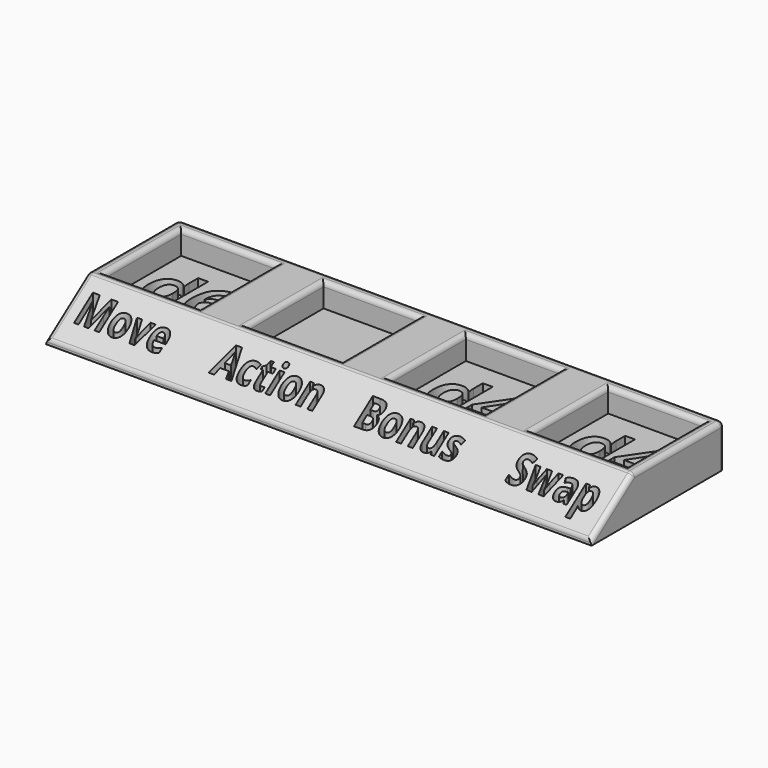
from build123d import *

# Parameters (mm, degrees)
F0_W           = 115
F0_H           = 35
F0_W_2         = 1.0340711806
F0_H_2         = 3.7912326389
F0_W_3         = 20
F0_H_3         = 20
F0_TEXT_SIZE   = 13.8888888889
F0_TEXT_SIZE_2 = 6.9444444444
F1_DEPTH       = 9
F2_DEPTH       = 5
F3_DEPTH       = 7.5
F4_DEPTH       = 8.5
F6_DEPTH       = 120
F7_T1_DEPTH    = 113
F7_T3_DEPTH    = 22.6748161864
F7_T5_DEPTH    = 15.7762866951
F7_T7_DEPTH    = 117.5461229585
F7_T9_DEPTH    = 15.7762866951
F7_T11_DEPTH   = 10.5
F7_T13_DEPTH   = 20
F7_T15_DEPTH   = 20
F7_T17_DEPTH   = 20
F7_T19_DEPTH   = 20
F7_T21_DEPTH   = 20
F7_S25_W       = 1
F7_S25_H       = 1
F7_T26_DEPTH   = 1
F7_S31_W       = 1
F7_S31_H       = 1
F7_T32_DEPTH   = 1
F7_T38_DEPTH   = 1
F7_T44_DEPTH   = 1
F7_T51_DEPTH   = 22.5
F7_T55_DEPTH   = 22.5
F7_T62_DEPTH   = 22.5
F7_T66_DEPTH   = 22.5
F7_T73_DEPTH   = 22.5
F7_T77_DEPTH   = 22.5
F7_T84_DEPTH   = 22.5
F7_T88_DEPTH   = 22.5
F7_T95_DEPTH   = 22.5
F7_T99_DEPTH   = 22.5
F7_T106_DEPTH  = 22.5
F7_T110_DEPTH  = 22.5
F7_T117_DEPTH  = 22.5
F7_T121_DEPTH  = 22.5
F7_T128_DEPTH  = 22.5
F7_T132_DEPTH  = 22.5
F7_T139_DEPTH  = 22.5
F7_T143_DEPTH  = 22.5
F7_T150_DEPTH  = 22.5
F7_T154_DEPTH  = 22.5
F7_T161_DEPTH  = 22.5
F7_T165_DEPTH  = 22.5
F7_T172_DEPTH  = 22.5
F7_T176_DEPTH  = 22.5
F7_T183_DEPTH  = 22.5
F7_T187_DEPTH  = 22.5
F7_T194_DEPTH  = 22.5
F7_T198_DEPTH  = 22.5
F7_T205_DEPTH  = 22.5
F7_T209_DEPTH  = 22.5
F7_T216_DEPTH  = 22.5
F7_T220_DEPTH  = 22.5


# Not quite as in the source:
# - a fillet or chamfer that OpenCascade refuses, or shapes differently, is made with other operations: its cross-section is extruded or revolved along the edge and cut away or added
# - Text() gives the source's letters only with a copy of the font that has no kerning and outlines rounded to 1/6400 em; it was checked with that copy


with BuildPart() as f1:
    # F0 (on Top) → F1 (new body)
    with BuildSketch(Plane.XY):
        with Locations((57.5, 17.5)):
            Rectangle(F0_W, F0_H)
        with BuildLine():
            Line((6.1859809028, 3.5), (5.2224392361, 3.5))
            Line((5.2224392361, 3.5), (4.0288628472, 7.3888888889))
            Line((4.0288628472, 7.3888888889), (3.9984809028, 7.3888888889))
            add(Edge.make_bspline(
                [(3.9984809028, 7.3888888889), (4.0635850694, 6.2029079861), (4.0635850694, 5.8057725694)],
                knots=[0, 0, 0, 1, 1, 1], degree=2))
            Line((4.0635850694, 5.8057725694), (4.0635850694, 3.5))
            Line((4.0635850694, 3.5), (3.1239149306, 3.5))
            Line((3.1239149306, 3.5), (3.1239149306, 8.4576822917))
            Line((3.1239149306, 8.4576822917), (4.5551215278, 8.4576822917))
            Line((4.5551215278, 8.4576822917), (5.7280815972, 4.6664496528))
            Line((5.7280815972, 4.6664496528), (5.7486979167, 4.6664496528))
            Line((5.7486979167, 4.6664496528), (6.9932725694, 8.4576822917))
            Line((6.9932725694, 8.4576822917), (8.4233940972, 8.4576822917))
            Line((8.4233940972, 8.4576822917), (8.4233940972, 3.5))
            Line((8.4233940972, 3.5), (7.4435763889, 3.5))
            Line((7.4435763889, 3.5), (7.4435763889, 5.8470052083))
            add(Edge.make_bspline(
                [(7.4435763889, 5.8470052083), (7.4435763889, 6.0130208333), (7.4490017361, 6.2300347222)],
                knots=[0, 0, 0, 1, 1, 1], degree=2))
            add(Edge.make_bspline(
                [(7.4490017361, 6.2300347222), (7.4544270833, 6.4470486111), (7.4945746528, 7.3823784722)],
                knots=[0, 0, 0, 1, 1, 1], degree=2))
            Line((7.4945746528, 7.3823784722), (7.4641927083, 7.3823784722))
            Line((7.4641927083, 7.3823784722), (6.1859809028, 3.5))
        make_face(mode=Mode.SUBTRACT)
        with BuildLine():
            add(Edge.make_bspline(
                [(12.8114149306, 6.4432508681), (13.0349392361, 5.9989149306), (13.0349392361, 5.4021267361)],
                knots=[0, 0, 0, 1, 1, 1], degree=2))
            add(Edge.make_bspline(
                [(13.0349392361, 5.4021267361), (13.0349392361, 4.4765625), (12.5466579861, 3.9541015625)],
                knots=[0, 0, 0, 1, 1, 1], degree=2))
            add(Edge.make_bspline(
                [(12.5466579861, 3.9541015625), (12.0583767361, 3.431640625), (11.1870659722, 3.431640625)],
                knots=[0, 0, 0, 1, 1, 1], degree=2))
            add(Edge.make_bspline(
                [(11.1870659722, 3.431640625), (10.6412760417, 3.431640625), (10.2240668403, 3.6708984375)],
                knots=[0, 0, 0, 1, 1, 1], degree=2))
            add(Edge.make_bspline(
                [(10.2240668403, 3.6708984375), (9.8068576389, 3.91015625), (9.5833333333, 4.3577473958)],
                knots=[0, 0, 0, 1, 1, 1], degree=2))
            add(Edge.make_bspline(
                [(9.5833333333, 4.3577473958), (9.3598090278, 4.8053385417), (9.3598090278, 5.4021267361)],
                knots=[0, 0, 0, 1, 1, 1], degree=2))
            add(Edge.make_bspline(
                [(9.3598090278, 5.4021267361), (9.3598090278, 6.3309461806), (9.8442925347, 6.8463541667)],
                knots=[0, 0, 0, 1, 1, 1], degree=2))
            add(Edge.make_bspline(
                [(9.8442925347, 6.8463541667), (10.3287760417, 7.3617621528), (11.2076822917, 7.3617621528)],
                knots=[0, 0, 0, 1, 1, 1], degree=2))
            add(Edge.make_bspline(
                [(11.2076822917, 7.3617621528), (11.7534722222, 7.3617621528), (12.1706814236, 7.1246744792)],
                knots=[0, 0, 0, 1, 1, 1], degree=2))
            add(Edge.make_bspline(
                [(12.1706814236, 7.1246744792), (12.587890625, 6.8875868056), (12.8114149306, 6.4432508681)],
                knots=[0, 0, 0, 1, 1, 1], degree=2))
        make_face(mode=Mode.SUBTRACT)
        with BuildLine():
            Line((15.8528645833, 3.5), (14.7916666667, 3.5))
            Line((14.7916666667, 3.5), (13.3474392361, 7.2912326389))
            Line((13.3474392361, 7.2912326389), (14.4292534722, 7.2912326389))
            Line((14.4292534722, 7.2912326389), (15.1616753472, 5.130859375))
            add(Edge.make_bspline(
                [(15.1616753472, 5.130859375), (15.283203125, 4.720703125), (15.3146701389, 4.3550347222)],
                knots=[0, 0, 0, 1, 1, 1], degree=2))
            Line((15.3146701389, 4.3550347222), (15.3342013889, 4.3550347222))
            add(Edge.make_bspline(
                [(15.3342013889, 4.3550347222), (15.3515625, 4.6805555556), (15.4871961806, 5.130859375)],
                knots=[0, 0, 0, 1, 1, 1], degree=2))
            Line((15.4871961806, 5.130859375), (16.2163628472, 7.2912326389))
            Line((16.2163628472, 7.2912326389), (17.2981770833, 7.2912326389))
            Line((17.2981770833, 7.2912326389), (15.8528645833, 3.5))
        make_face(mode=Mode.SUBTRACT)
        with BuildLine():
            add(Edge.make_bspline(
                [(20.3092447917, 3.4978298611), (20.0010850694, 3.431640625), (19.5562065972, 3.431640625)],
                knots=[0, 0, 0, 1, 1, 1], degree=2))
            add(Edge.make_bspline(
                [(19.5562065972, 3.431640625), (18.6414930556, 3.431640625), (18.1260850694, 3.9372829861)],
                knots=[0, 0, 0, 1, 1, 1], degree=2))
            add(Edge.make_bspline(
                [(18.1260850694, 3.9372829861), (17.6106770833, 4.4429253472), (17.6106770833, 5.3684895833)],
                knots=[0, 0, 0, 1, 1, 1], degree=2))
            add(Edge.make_bspline(
                [(17.6106770833, 5.3684895833), (17.6106770833, 6.3211805556), (18.0870225694, 6.8414713542)],
                knots=[0, 0, 0, 1, 1, 1], degree=2))
            add(Edge.make_bspline(
                [(18.0870225694, 6.8414713542), (18.5633680556, 7.3617621528), (19.404296875, 7.3617621528)],
                knots=[0, 0, 0, 1, 1, 1], degree=2))
            add(Edge.make_bspline(
                [(19.404296875, 7.3617621528), (20.2072482639, 7.3617621528), (20.6548394097, 6.9044053819)],
                knots=[0, 0, 0, 1, 1, 1], degree=2))
            add(Edge.make_bspline(
                [(20.6548394097, 6.9044053819), (21.1024305556, 6.4470486111), (21.1024305556, 5.6397569444)],
                knots=[0, 0, 0, 1, 1, 1], degree=2))
            Line((21.1024305556, 5.6397569444), (21.1024305556, 5.1373697917))
            Line((21.1024305556, 5.1373697917), (18.6577690972, 5.1373697917))
            add(Edge.make_bspline(
                [(18.6577690972, 5.1373697917), (18.6751302083, 4.6968315972), (18.9192708333, 4.4494357639)],
                knots=[0, 0, 0, 1, 1, 1], degree=2))
            add(Edge.make_bspline(
                [(18.9192708333, 4.4494357639), (19.1634114583, 4.2020399306), (19.6039496528, 4.2020399306)],
                knots=[0, 0, 0, 1, 1, 1], degree=2))
            add(Edge.make_bspline(
                [(19.6039496528, 4.2020399306), (19.9468315972, 4.2020399306), (20.2517361111, 4.2731119792)],
                knots=[0, 0, 0, 1, 1, 1], degree=2))
            add(Edge.make_bspline(
                [(20.2517361111, 4.2731119792), (20.556640625, 4.3441840278), (20.888671875, 4.5004340278)],
                knots=[0, 0, 0, 1, 1, 1], degree=2))
            Line((20.888671875, 4.5004340278), (20.888671875, 3.6996527778))
            add(Edge.make_bspline(
                [(20.888671875, 3.6996527778), (20.6174045139, 3.5640190972), (20.3092447917, 3.4978298611)],
                knots=[0, 0, 0, 1, 1, 1], degree=2))
        make_face(mode=Mode.SUBTRACT)
        Polygon((36.2916666667, 3.5), (35.1588541667, 3.5), (34.7996961806, 4.6805555556), (32.9919704861, 4.6805555556), (32.6328125, 3.5), (31.5, 3.5), (33.2502170139, 8.4782986111), (34.5349392361, 8.4782986111), align=None, mode=Mode.SUBTRACT)
        with BuildLine():
            add(Edge.make_bspline(
                [(39.01953125, 3.4929470486), (38.7634548611, 3.431640625), (38.3739149306, 3.431640625)],
                knots=[0, 0, 0, 1, 1, 1], degree=2))
            add(Edge.make_bspline(
                [(38.3739149306, 3.431640625), (36.6041666667, 3.431640625), (36.6041666667, 5.375)],
                knots=[0, 0, 0, 1, 1, 1], degree=2))
            add(Edge.make_bspline(
                [(36.6041666667, 5.375), (36.6041666667, 6.341796875), (37.0853949653, 6.8517795139)],
                knots=[0, 0, 0, 1, 1, 1], degree=2))
            add(Edge.make_bspline(
                [(37.0853949653, 6.8517795139), (37.5666232639, 7.3617621528), (38.4650607639, 7.3617621528)],
                knots=[0, 0, 0, 1, 1, 1], degree=2))
            add(Edge.make_bspline(
                [(38.4650607639, 7.3617621528), (39.1226128472, 7.3617621528), (39.6456163194, 7.1046006944)],
                knots=[0, 0, 0, 1, 1, 1], degree=2))
            Line((39.6456163194, 7.1046006944), (39.3396267361, 6.3038194444))
            add(Edge.make_bspline(
                [(39.3396267361, 6.3038194444), (39.0954861111, 6.4025607639), (38.8855251736, 6.4654947917)],
                knots=[0, 0, 0, 1, 1, 1], degree=2))
            add(Edge.make_bspline(
                [(38.8855251736, 6.4654947917), (38.6755642361, 6.5284288194), (38.4650607639, 6.5284288194)],
                knots=[0, 0, 0, 1, 1, 1], degree=2))
            add(Edge.make_bspline(
                [(38.4650607639, 6.5284288194), (37.6577690972, 6.5284288194), (37.6577690972, 5.3815104167)],
                knots=[0, 0, 0, 1, 1, 1], degree=2))
            add(Edge.make_bspline(
                [(37.6577690972, 5.3815104167), (37.6577690972, 4.2693142361), (38.4650607639, 4.2693142361)],
                knots=[0, 0, 0, 1, 1, 1], degree=2))
            add(Edge.make_bspline(
                [(38.4650607639, 4.2693142361), (38.7634548611, 4.2693142361), (39.0179036458, 4.3490668403)],
                knots=[0, 0, 0, 1, 1, 1], degree=2))
            add(Edge.make_bspline(
                [(39.0179036458, 4.3490668403), (39.2723524306, 4.4288194444), (39.5262586806, 4.5991753472)],
                knots=[0, 0, 0, 1, 1, 1], degree=2))
            Line((39.5262586806, 4.5991753472), (39.5262586806, 3.7137586806))
            add(Edge.make_bspline(
                [(39.5262586806, 3.7137586806), (39.2756076389, 3.5542534722), (39.01953125, 3.4929470486)],
                knots=[0, 0, 0, 1, 1, 1], degree=2))
        make_face(mode=Mode.SUBTRACT)
        with BuildLine():
            add(Edge.make_bspline(
                [(41.6746961806, 4.3615451389), (41.7983940972, 4.2562934028), (42.0023871528, 4.2562934028)],
                knots=[0, 0, 0, 1, 1, 1], degree=2))
            add(Edge.make_bspline(
                [(42.0023871528, 4.2562934028), (42.2736545139, 4.2562934028), (42.6534288194, 4.3745659722)],
                knots=[0, 0, 0, 1, 1, 1], degree=2))
            Line((42.6534288194, 4.3745659722), (42.6534288194, 3.6052517361))
            add(Edge.make_bspline(
                [(42.6534288194, 3.6052517361), (42.2671440972, 3.431640625), (41.7039930556, 3.431640625)],
                knots=[0, 0, 0, 1, 1, 1], degree=2))
            add(Edge.make_bspline(
                [(41.7039930556, 3.431640625), (41.0833333333, 3.431640625), (40.8001302083, 3.7457682292)],
                knots=[0, 0, 0, 1, 1, 1], degree=2))
            add(Edge.make_bspline(
                [(40.8001302083, 3.7457682292), (40.5169270833, 4.0598958333), (40.5169270833, 4.6870659722)],
                knots=[0, 0, 0, 1, 1, 1], degree=2))
            Line((40.5169270833, 4.6870659722), (40.5169270833, 6.5143229167))
            Line((40.5169270833, 6.5143229167), (40.0221354167, 6.5143229167))
            Line((40.0221354167, 6.5143229167), (40.0221354167, 6.9516059028))
            Line((40.0221354167, 6.9516059028), (40.591796875, 7.2977430556))
            Line((40.591796875, 7.2977430556), (40.8901909722, 8.0985243056))
            Line((40.8901909722, 8.0985243056), (41.5509982639, 8.0985243056))
            Line((41.5509982639, 8.0985243056), (41.5509982639, 7.2912326389))
            Line((41.5509982639, 7.2912326389), (42.6121961806, 7.2912326389))
            Line((42.6121961806, 7.2912326389), (42.6121961806, 6.5143229167))
            Line((42.6121961806, 6.5143229167), (41.5509982639, 6.5143229167))
            Line((41.5509982639, 6.5143229167), (41.5509982639, 4.6870659722))
            add(Edge.make_bspline(
                [(41.5509982639, 4.6870659722), (41.5509982639, 4.466796875), (41.6746961806, 4.3615451389)],
                knots=[0, 0, 0, 1, 1, 1], degree=2))
        make_face(mode=Mode.SUBTRACT)
        with Locations((43.9365234375, 5.3956163194)):
            Rectangle(F0_W_2, F0_H_2, mode=Mode.SUBTRACT)
        with BuildLine():
            add(Edge.make_bspline(
                [(48.7601996528, 6.4432508681), (48.9837239583, 5.9989149306), (48.9837239583, 5.4021267361)],
                knots=[0, 0, 0, 1, 1, 1], degree=2))
            add(Edge.make_bspline(
                [(48.9837239583, 5.4021267361), (48.9837239583, 4.4765625), (48.4954427083, 3.9541015625)],
                knots=[0, 0, 0, 1, 1, 1], degree=2))
            add(Edge.make_bspline(
                [(48.4954427083, 3.9541015625), (48.0071614583, 3.431640625), (47.1358506944, 3.431640625)],
                knots=[0, 0, 0, 1, 1, 1], degree=2))
            add(Edge.make_bspline(
                [(47.1358506944, 3.431640625), (46.5900607639, 3.431640625), (46.1728515625, 3.6708984375)],
                knots=[0, 0, 0, 1, 1, 1], degree=2))
            add(Edge.make_bspline(
                [(46.1728515625, 3.6708984375), (45.7556423611, 3.91015625), (45.5321180556, 4.3577473958)],
                knots=[0, 0, 0, 1, 1, 1], degree=2))
            add(Edge.make_bspline(
                [(45.5321180556, 4.3577473958), (45.30859375, 4.8053385417), (45.30859375, 5.4021267361)],
                knots=[0, 0, 0, 1, 1, 1], degree=2))
            add(Edge.make_bspline(
                [(45.30859375, 5.4021267361), (45.30859375, 6.3309461806), (45.7930772569, 6.8463541667)],
                knots=[0, 0, 0, 1, 1, 1], degree=2))
            add(Edge.make_bspline(
                [(45.7930772569, 6.8463541667), (46.2775607639, 7.3617621528), (47.1564670139, 7.3617621528)],
                knots=[0, 0, 0, 1, 1, 1], degree=2))
            add(Edge.make_bspline(
                [(47.1564670139, 7.3617621528), (47.7022569444, 7.3617621528), (48.1194661458, 7.1246744792)],
                knots=[0, 0, 0, 1, 1, 1], degree=2))
            add(Edge.make_bspline(
                [(48.1194661458, 7.1246744792), (48.5366753472, 6.8875868056), (48.7601996528, 6.4432508681)],
                knots=[0, 0, 0, 1, 1, 1], degree=2))
        make_face(mode=Mode.SUBTRACT)
        with BuildLine():
            Line((53.3381076389, 5.9717881944), (53.3381076389, 3.5))
            Line((53.3381076389, 3.5), (52.3040364583, 3.5))
            Line((52.3040364583, 3.5), (52.3040364583, 5.7146267361))
            add(Edge.make_bspline(
                [(52.3040364583, 5.7146267361), (52.3040364583, 6.1247829861), (52.1580946181, 6.3298611111)],
                knots=[0, 0, 0, 1, 1, 1], degree=2))
            add(Edge.make_bspline(
                [(52.1580946181, 6.3298611111), (52.0121527778, 6.5349392361), (51.6931423611, 6.5349392361)],
                knots=[0, 0, 0, 1, 1, 1], degree=2))
            add(Edge.make_bspline(
                [(51.6931423611, 6.5349392361), (51.2591145833, 6.5349392361), (51.0659722222, 6.2452256944)],
                knots=[0, 0, 0, 1, 1, 1], degree=2))
            add(Edge.make_bspline(
                [(51.0659722222, 6.2452256944), (50.8728298611, 5.9555121528), (50.8728298611, 5.2838541667)],
                knots=[0, 0, 0, 1, 1, 1], degree=2))
            Line((50.8728298611, 5.2838541667), (50.8728298611, 3.5))
            Line((50.8728298611, 3.5), (49.8387586806, 3.5))
            Line((49.8387586806, 3.5), (49.8387586806, 7.2912326389))
            Line((49.8387586806, 7.2912326389), (50.6286892361, 7.2912326389))
            Line((50.6286892361, 7.2912326389), (50.767578125, 6.8062065972))
            Line((50.767578125, 6.8062065972), (50.8250868056, 6.8062065972))
            add(Edge.make_bspline(
                [(50.8250868056, 6.8062065972), (50.9986979167, 7.0807291667), (51.3019748264, 7.2212456597)],
                knots=[0, 0, 0, 1, 1, 1], degree=2))
            add(Edge.make_bspline(
                [(51.3019748264, 7.2212456597), (51.6052517361, 7.3617621528), (51.9915364583, 7.3617621528)],
                knots=[0, 0, 0, 1, 1, 1], degree=2))
            add(Edge.make_bspline(
                [(51.9915364583, 7.3617621528), (52.6534288194, 7.3617621528), (52.9957682292, 7.0042317708)],
                knots=[0, 0, 0, 1, 1, 1], degree=2))
            add(Edge.make_bspline(
                [(52.9957682292, 7.0042317708), (53.3381076389, 6.6467013889), (53.3381076389, 5.9717881944)],
                knots=[0, 0, 0, 1, 1, 1], degree=2))
        make_face(mode=Mode.SUBTRACT)
        with BuildLine():
            add(Edge.make_bspline(
                [(43.9381510417, 7.7621527778), (43.375, 7.7621527778), (43.375, 8.2710503472)],
                knots=[0, 0, 0, 1, 1, 1], degree=2))
            add(Edge.make_bspline(
                [(43.375, 8.2710503472), (43.375, 8.7766927083), (43.9381510417, 8.7766927083)],
                knots=[0, 0, 0, 1, 1, 1], degree=2))
            add(Edge.make_bspline(
                [(43.9381510417, 8.7766927083), (44.5013020833, 8.7766927083), (44.5013020833, 8.2710503472)],
                knots=[0, 0, 0, 1, 1, 1], degree=2))
            add(Edge.make_bspline(
                [(44.5013020833, 8.2710503472), (44.5013020833, 8.0301649306), (44.3607855903, 7.8961588542)],
                knots=[0, 0, 0, 1, 1, 1], degree=2))
            add(Edge.make_bspline(
                [(44.3607855903, 7.8961588542), (44.2202690972, 7.7621527778), (43.9381510417, 7.7621527778)],
                knots=[0, 0, 0, 1, 1, 1], degree=2))
        make_face(mode=Mode.SUBTRACT)
        with BuildLine():
            Line((62.1239149306, 3.5), (62.1239149306, 8.4576822917))
            Line((62.1239149306, 8.4576822917), (63.6668836806, 8.4576822917))
            add(Edge.make_bspline(
                [(63.6668836806, 8.4576822917), (64.7215711806, 8.4576822917), (65.1979166667, 8.1576605903)],
                knots=[0, 0, 0, 1, 1, 1], degree=2))
            add(Edge.make_bspline(
                [(65.1979166667, 8.1576605903), (65.6742621528, 7.8576388889), (65.6742621528, 7.2033420139)],
                knots=[0, 0, 0, 1, 1, 1], degree=2))
            add(Edge.make_bspline(
                [(65.6742621528, 7.2033420139), (65.6742621528, 6.7584635417), (65.4659288194, 6.4736328125)],
                knots=[0, 0, 0, 1, 1, 1], degree=2))
            add(Edge.make_bspline(
                [(65.4659288194, 6.4736328125), (65.2575954861, 6.1888020833), (64.9114583333, 6.1312934028)],
                knots=[0, 0, 0, 1, 1, 1], degree=2))
            Line((64.9114583333, 6.1312934028), (64.9114583333, 6.09765625))
            add(Edge.make_bspline(
                [(64.9114583333, 6.09765625), (65.3823784722, 5.9924045139), (65.5912543403, 5.7043185764)],
                knots=[0, 0, 0, 1, 1, 1], degree=2))
            add(Edge.make_bspline(
                [(65.5912543403, 5.7043185764), (65.8001302083, 5.4162326389), (65.8001302083, 4.9377170139)],
                knots=[0, 0, 0, 1, 1, 1], degree=2))
            add(Edge.make_bspline(
                [(65.8001302083, 4.9377170139), (65.8001302083, 4.2595486111), (65.3096788194, 3.8797743056)],
                knots=[0, 0, 0, 1, 1, 1], degree=2))
            add(Edge.make_bspline(
                [(65.3096788194, 3.8797743056), (64.8192274306, 3.5), (63.9782986111, 3.5)],
                knots=[0, 0, 0, 1, 1, 1], degree=2))
            Line((63.9782986111, 3.5), (62.1239149306, 3.5))
        make_face(mode=Mode.SUBTRACT)
        with BuildLine():
            add(Edge.make_bspline(
                [(69.9299045139, 6.4432508681), (70.1534288194, 5.9989149306), (70.1534288194, 5.4021267361)],
                knots=[0, 0, 0, 1, 1, 1], degree=2))
            add(Edge.make_bspline(
                [(70.1534288194, 5.4021267361), (70.1534288194, 4.4765625), (69.6651475694, 3.9541015625)],
                knots=[0, 0, 0, 1, 1, 1], degree=2))
            add(Edge.make_bspline(
                [(69.6651475694, 3.9541015625), (69.1768663194, 3.431640625), (68.3055555556, 3.431640625)],
                knots=[0, 0, 0, 1, 1, 1], degree=2))
            add(Edge.make_bspline(
                [(68.3055555556, 3.431640625), (67.759765625, 3.431640625), (67.3425564236, 3.6708984375)],
                knots=[0, 0, 0, 1, 1, 1], degree=2))
            add(Edge.make_bspline(
                [(67.3425564236, 3.6708984375), (66.9253472222, 3.91015625), (66.7018229167, 4.3577473958)],
                knots=[0, 0, 0, 1, 1, 1], degree=2))
            add(Edge.make_bspline(
                [(66.7018229167, 4.3577473958), (66.4782986111, 4.8053385417), (66.4782986111, 5.4021267361)],
                knots=[0, 0, 0, 1, 1, 1], degree=2))
            add(Edge.make_bspline(
                [(66.4782986111, 5.4021267361), (66.4782986111, 6.3309461806), (66.9627821181, 6.8463541667)],
                knots=[0, 0, 0, 1, 1, 1], degree=2))
            add(Edge.make_bspline(
                [(66.9627821181, 6.8463541667), (67.447265625, 7.3617621528), (68.326171875, 7.3617621528)],
                knots=[0, 0, 0, 1, 1, 1], degree=2))
            add(Edge.make_bspline(
                [(68.326171875, 7.3617621528), (68.8719618056, 7.3617621528), (69.2891710069, 7.1246744792)],
                knots=[0, 0, 0, 1, 1, 1], degree=2))
            add(Edge.make_bspline(
                [(69.2891710069, 7.1246744792), (69.7063802083, 6.8875868056), (69.9299045139, 6.4432508681)],
                knots=[0, 0, 0, 1, 1, 1], degree=2))
        make_face(mode=Mode.SUBTRACT)
        with BuildLine():
            Line((74.5078125, 5.9717881944), (74.5078125, 3.5))
            Line((74.5078125, 3.5), (73.4737413194, 3.5))
            Line((73.4737413194, 3.5), (73.4737413194, 5.7146267361))
            add(Edge.make_bspline(
                [(73.4737413194, 5.7146267361), (73.4737413194, 6.1247829861), (73.3277994792, 6.3298611111)],
                knots=[0, 0, 0, 1, 1, 1], degree=2))
            add(Edge.make_bspline(
                [(73.3277994792, 6.3298611111), (73.1818576389, 6.5349392361), (72.8628472222, 6.5349392361)],
                knots=[0, 0, 0, 1, 1, 1], degree=2))
            add(Edge.make_bspline(
                [(72.8628472222, 6.5349392361), (72.4288194444, 6.5349392361), (72.2356770833, 6.2452256944)],
                knots=[0, 0, 0, 1, 1, 1], degree=2))
            add(Edge.make_bspline(
                [(72.2356770833, 6.2452256944), (72.0425347222, 5.9555121528), (72.0425347222, 5.2838541667)],
                knots=[0, 0, 0, 1, 1, 1], degree=2))
            Line((72.0425347222, 5.2838541667), (72.0425347222, 3.5))
            Line((72.0425347222, 3.5), (71.0084635417, 3.5))
            Line((71.0084635417, 3.5), (71.0084635417, 7.2912326389))
            Line((71.0084635417, 7.2912326389), (71.7983940972, 7.2912326389))
            Line((71.7983940972, 7.2912326389), (71.9372829861, 6.8062065972))
            Line((71.9372829861, 6.8062065972), (71.9947916667, 6.8062065972))
            add(Edge.make_bspline(
                [(71.9947916667, 6.8062065972), (72.1684027778, 7.0807291667), (72.4716796875, 7.2212456597)],
                knots=[0, 0, 0, 1, 1, 1], degree=2))
            add(Edge.make_bspline(
                [(72.4716796875, 7.2212456597), (72.7749565972, 7.3617621528), (73.1612413194, 7.3617621528)],
                knots=[0, 0, 0, 1, 1, 1], degree=2))
            add(Edge.make_bspline(
                [(73.1612413194, 7.3617621528), (73.8231336806, 7.3617621528), (74.1654730903, 7.0042317708)],
                knots=[0, 0, 0, 1, 1, 1], degree=2))
            add(Edge.make_bspline(
                [(74.1654730903, 7.0042317708), (74.5078125, 6.6467013889), (74.5078125, 5.9717881944)],
                knots=[0, 0, 0, 1, 1, 1], degree=2))
        make_face(mode=Mode.SUBTRACT)
        with BuildLine():
            Line((79.0509982639, 3.5), (78.2578125, 3.5))
            Line((78.2578125, 3.5), (78.1189236111, 3.9850260417))
            Line((78.1189236111, 3.9850260417), (78.0646701389, 3.9850260417))
            add(Edge.make_bspline(
                [(78.0646701389, 3.9850260417), (77.8986545139, 3.7202690972), (77.5932074653, 3.5759548611)],
                knots=[0, 0, 0, 1, 1, 1], degree=2))
            add(Edge.make_bspline(
                [(77.5932074653, 3.5759548611), (77.2877604167, 3.431640625), (76.8982204861, 3.431640625)],
                knots=[0, 0, 0, 1, 1, 1], degree=2))
            add(Edge.make_bspline(
                [(76.8982204861, 3.431640625), (76.2298177083, 3.431640625), (75.8907335069, 3.7897135417)],
                knots=[0, 0, 0, 1, 1, 1], degree=2))
            add(Edge.make_bspline(
                [(75.8907335069, 3.7897135417), (75.5516493056, 4.1477864583), (75.5516493056, 4.8194444444)],
                knots=[0, 0, 0, 1, 1, 1], degree=2))
            Line((75.5516493056, 4.8194444444), (75.5516493056, 7.2912326389))
            Line((75.5516493056, 7.2912326389), (76.5857204861, 7.2912326389))
            Line((76.5857204861, 7.2912326389), (76.5857204861, 5.0766059028))
            add(Edge.make_bspline(
                [(76.5857204861, 5.0766059028), (76.5857204861, 4.6664496528), (76.7316623264, 4.4613715278)],
                knots=[0, 0, 0, 1, 1, 1], degree=2))
            add(Edge.make_bspline(
                [(76.7316623264, 4.4613715278), (76.8776041667, 4.2562934028), (77.1966145833, 4.2562934028)],
                knots=[0, 0, 0, 1, 1, 1], degree=2))
            add(Edge.make_bspline(
                [(77.1966145833, 4.2562934028), (77.6306423611, 4.2562934028), (77.8237847222, 4.5460069444)],
                knots=[0, 0, 0, 1, 1, 1], degree=2))
            add(Edge.make_bspline(
                [(77.8237847222, 4.5460069444), (78.0169270833, 4.8357204861), (78.0169270833, 5.5073784722)],
                knots=[0, 0, 0, 1, 1, 1], degree=2))
            Line((78.0169270833, 5.5073784722), (78.0169270833, 7.2912326389))
            Line((78.0169270833, 7.2912326389), (79.0509982639, 7.2912326389))
            Line((79.0509982639, 7.2912326389), (79.0509982639, 3.5))
        make_face(mode=Mode.SUBTRACT)
        with BuildLine():
            add(Edge.make_bspline(
                [(82.6827256944, 5.1107855903), (82.7814670139, 4.9073350694), (82.7814670139, 4.6263020833)],
                knots=[0, 0, 0, 1, 1, 1], degree=2))
            add(Edge.make_bspline(
                [(82.7814670139, 4.6263020833), (82.7814670139, 4.0425347222), (82.3761935764, 3.7370876736)],
                knots=[0, 0, 0, 1, 1, 1], degree=2))
            add(Edge.make_bspline(
                [(82.3761935764, 3.7370876736), (81.9709201389, 3.431640625), (81.1636284722, 3.431640625)],
                knots=[0, 0, 0, 1, 1, 1], degree=2))
            add(Edge.make_bspline(
                [(81.1636284722, 3.431640625), (80.7502170139, 3.431640625), (80.4583333333, 3.4880642361)],
                knots=[0, 0, 0, 1, 1, 1], degree=2))
            add(Edge.make_bspline(
                [(80.4583333333, 3.4880642361), (80.1664496528, 3.5444878472), (79.9125434028, 3.6529947917)],
                knots=[0, 0, 0, 1, 1, 1], degree=2))
            Line((79.9125434028, 3.6529947917), (79.9125434028, 4.5069444444))
            add(Edge.make_bspline(
                [(79.9125434028, 4.5069444444), (80.2000868056, 4.3713107639), (80.5614149306, 4.2796223958)],
                knots=[0, 0, 0, 1, 1, 1], degree=2))
            add(Edge.make_bspline(
                [(80.5614149306, 4.2796223958), (80.9227430556, 4.1879340278), (81.197265625, 4.1879340278)],
                knots=[0, 0, 0, 1, 1, 1], degree=2))
            add(Edge.make_bspline(
                [(81.197265625, 4.1879340278), (81.7604166667, 4.1879340278), (81.7604166667, 4.5134548611)],
                knots=[0, 0, 0, 1, 1, 1], degree=2))
            add(Edge.make_bspline(
                [(81.7604166667, 4.5134548611), (81.7604166667, 4.6360677083), (81.685546875, 4.7125651042)],
                knots=[0, 0, 0, 1, 1, 1], degree=2))
            add(Edge.make_bspline(
                [(81.685546875, 4.7125651042), (81.6106770833, 4.7890625), (81.4278428819, 4.8856336806)],
                knots=[0, 0, 0, 1, 1, 1], degree=2))
            add(Edge.make_bspline(
                [(81.4278428819, 4.8856336806), (81.2450086806, 4.9822048611), (80.9401041667, 5.1102430556)],
                knots=[0, 0, 0, 1, 1, 1], degree=2))
            add(Edge.make_bspline(
                [(80.9401041667, 5.1102430556), (80.5028211806, 5.2936197917), (80.2972005208, 5.4498697917)],
                knots=[0, 0, 0, 1, 1, 1], degree=2))
            add(Edge.make_bspline(
                [(80.2972005208, 5.4498697917), (80.0915798611, 5.6061197917), (79.9988064236, 5.8079427083)],
                knots=[0, 0, 0, 1, 1, 1], degree=2))
            add(Edge.make_bspline(
                [(79.9988064236, 5.8079427083), (79.9060329861, 6.009765625), (79.9060329861, 6.3038194444)],
                knots=[0, 0, 0, 1, 1, 1], degree=2))
            add(Edge.make_bspline(
                [(79.9060329861, 6.3038194444), (79.9060329861, 6.8094618056), (80.2972005208, 7.0856119792)],
                knots=[0, 0, 0, 1, 1, 1], degree=2))
            add(Edge.make_bspline(
                [(80.2972005208, 7.0856119792), (80.6883680556, 7.3617621528), (81.4077690972, 7.3617621528)],
                knots=[0, 0, 0, 1, 1, 1], degree=2))
            add(Edge.make_bspline(
                [(81.4077690972, 7.3617621528), (82.0924479167, 7.3617621528), (82.740234375, 7.0633680556)],
                knots=[0, 0, 0, 1, 1, 1], degree=2))
            Line((82.740234375, 7.0633680556), (82.4288194444, 6.3179253472))
            add(Edge.make_bspline(
                [(82.4288194444, 6.3179253472), (82.1434461806, 6.439453125), (81.8960503472, 6.517578125)],
                knots=[0, 0, 0, 1, 1, 1], degree=2))
            add(Edge.make_bspline(
                [(81.8960503472, 6.517578125), (81.6486545139, 6.595703125), (81.3904079861, 6.595703125)],
                knots=[0, 0, 0, 1, 1, 1], degree=2))
            add(Edge.make_bspline(
                [(81.3904079861, 6.595703125), (80.9325086806, 6.595703125), (80.9325086806, 6.3483072917)],
                knots=[0, 0, 0, 1, 1, 1], degree=2))
            add(Edge.make_bspline(
                [(80.9325086806, 6.3483072917), (80.9325086806, 6.2094184028), (81.080078125, 6.107421875)],
                knots=[0, 0, 0, 1, 1, 1], degree=2))
            add(Edge.make_bspline(
                [(81.080078125, 6.107421875), (81.2276475694, 6.0054253472), (81.7267795139, 5.8057725694)],
                knots=[0, 0, 0, 1, 1, 1], degree=2))
            add(Edge.make_bspline(
                [(81.7267795139, 5.8057725694), (82.1705729167, 5.6256510417), (82.3772786458, 5.4699435764)],
                knots=[0, 0, 0, 1, 1, 1], degree=2))
            add(Edge.make_bspline(
                [(82.3772786458, 5.4699435764), (82.583984375, 5.3142361111), (82.6827256944, 5.1107855903)],
                knots=[0, 0, 0, 1, 1, 1], degree=2))
        make_face(mode=Mode.SUBTRACT)
        with BuildLine():
            Line((102.1089409722, 3.5), (100.9837239583, 3.5))
            Line((100.9837239583, 3.5), (100.6918402778, 4.8259548611))
            Line((100.6918402778, 4.8259548611), (100.2990451389, 6.5013020833))
            Line((100.2990451389, 6.5013020833), (100.2751736111, 6.5013020833))
            Line((100.2751736111, 6.5013020833), (99.5828993056, 3.5))
            Line((99.5828993056, 3.5), (98.470703125, 3.5))
            Line((98.470703125, 3.5), (97.3932291667, 7.2912326389))
            Line((97.3932291667, 7.2912326389), (98.4240451389, 7.2912326389))
            Line((98.4240451389, 7.2912326389), (98.861328125, 5.6126302083))
            add(Edge.make_bspline(
                [(98.861328125, 5.6126302083), (98.9665798611, 5.1612413194), (99.0750868056, 4.3680555556)],
                knots=[0, 0, 0, 1, 1, 1], degree=2))
            Line((99.0750868056, 4.3680555556), (99.0946180556, 4.3680555556))
            add(Edge.make_bspline(
                [(99.0946180556, 4.3680555556), (99.1087239583, 4.6263020833), (99.2139756944, 5.1851128472)],
                knots=[0, 0, 0, 1, 1, 1], degree=2))
            Line((99.2139756944, 5.1851128472), (99.2682291667, 5.4737413194))
            Line((99.2682291667, 5.4737413194), (99.7358940972, 7.2912326389))
            Line((99.7358940972, 7.2912326389), (100.8752170139, 7.2912326389))
            Line((100.8752170139, 7.2912326389), (101.3190104167, 5.4737413194))
            add(Edge.make_bspline(
                [(101.3190104167, 5.4737413194), (101.3331163194, 5.3988715278), (101.3618706597, 5.2529296875)],
                knots=[0, 0, 0, 1, 1, 1], degree=2))
            add(Edge.make_bspline(
                [(101.3618706597, 5.2529296875), (101.390625, 5.1069878472), (101.4177517361, 4.9425998264)],
                knots=[0, 0, 0, 1, 1, 1], degree=2))
            add(Edge.make_bspline(
                [(101.4177517361, 4.9425998264), (101.4448784722, 4.7782118056), (101.4671223958, 4.6208767361)],
                knots=[0, 0, 0, 1, 1, 1], degree=2))
            add(Edge.make_bspline(
                [(101.4671223958, 4.6208767361), (101.4893663194, 4.4635416667), (101.4926215278, 4.3680555556)],
                knots=[0, 0, 0, 1, 1, 1], degree=2))
            Line((101.4926215278, 4.3680555556), (101.5121527778, 4.3680555556))
            add(Edge.make_bspline(
                [(101.5121527778, 4.3680555556), (101.5436197917, 4.6121961806), (101.6212022569, 5.0375434028)],
                knots=[0, 0, 0, 1, 1, 1], degree=2))
            add(Edge.make_bspline(
                [(101.6212022569, 5.0375434028), (101.6987847222, 5.462890625), (101.7335069444, 5.6126302083)],
                knots=[0, 0, 0, 1, 1, 1], degree=2))
            Line((101.7335069444, 5.6126302083), (102.1870659722, 7.2912326389))
            Line((102.1870659722, 7.2912326389), (103.2016059028, 7.2912326389))
            Line((103.2016059028, 7.2912326389), (102.1089409722, 3.5))
        make_face(mode=Mode.SUBTRACT)
        with BuildLine():
            add(Edge.make_bspline(
                [(96.7926432292, 5.6956380208), (97.0503472222, 5.3619791667), (97.0503472222, 4.876953125)],
                knots=[0, 0, 0, 1, 1, 1], degree=2))
            add(Edge.make_bspline(
                [(97.0503472222, 4.876953125), (97.0503472222, 4.2052951389), (96.5669487847, 3.8184678819)],
                knots=[0, 0, 0, 1, 1, 1], degree=2))
            add(Edge.make_bspline(
                [(96.5669487847, 3.8184678819), (96.0835503472, 3.431640625), (95.2230902778, 3.431640625)],
                knots=[0, 0, 0, 1, 1, 1], degree=2))
            add(Edge.make_bspline(
                [(95.2230902778, 3.431640625), (94.4288194444, 3.431640625), (93.8190104167, 3.7311197917)],
                knots=[0, 0, 0, 1, 1, 1], degree=2))
            Line((93.8190104167, 3.7311197917), (93.8190104167, 4.7076822917))
            add(Edge.make_bspline(
                [(93.8190104167, 4.7076822917), (94.3203125, 4.4830729167), (94.6680772569, 4.3919270833)],
                knots=[0, 0, 0, 1, 1, 1], degree=2))
            add(Edge.make_bspline(
                [(94.6680772569, 4.3919270833), (95.0158420139, 4.30078125), (95.3044704861, 4.30078125)],
                knots=[0, 0, 0, 1, 1, 1], degree=2))
            add(Edge.make_bspline(
                [(95.3044704861, 4.30078125), (95.6495225694, 4.30078125), (95.8345269097, 4.4326171875)],
                knots=[0, 0, 0, 1, 1, 1], degree=2))
            add(Edge.make_bspline(
                [(95.8345269097, 4.4326171875), (96.01953125, 4.564453125), (96.01953125, 4.8259548611)],
                knots=[0, 0, 0, 1, 1, 1], degree=2))
            add(Edge.make_bspline(
                [(96.01953125, 4.8259548611), (96.01953125, 4.9713541667), (95.9381510417, 5.0852864583)],
                knots=[0, 0, 0, 1, 1, 1], degree=2))
            add(Edge.make_bspline(
                [(95.9381510417, 5.0852864583), (95.8567708333, 5.19921875), (95.6988932292, 5.3039279514)],
                knots=[0, 0, 0, 1, 1, 1], degree=2))
            add(Edge.make_bspline(
                [(95.6988932292, 5.3039279514), (95.541015625, 5.4086371528), (95.0559895833, 5.6397569444)],
                knots=[0, 0, 0, 1, 1, 1], degree=2))
            add(Edge.make_bspline(
                [(95.0559895833, 5.6397569444), (94.6024305556, 5.853515625), (94.3751085069, 6.0499131944)],
                knots=[0, 0, 0, 1, 1, 1], degree=2))
            add(Edge.make_bspline(
                [(94.3751085069, 6.0499131944), (94.1477864583, 6.2463107639), (94.0121527778, 6.5078125)],
                knots=[0, 0, 0, 1, 1, 1], degree=2))
            add(Edge.make_bspline(
                [(94.0121527778, 6.5078125), (93.8765190972, 6.7693142361), (93.8765190972, 7.1176215278)],
                knots=[0, 0, 0, 1, 1, 1], degree=2))
            add(Edge.make_bspline(
                [(93.8765190972, 7.1176215278), (93.8765190972, 7.7762586806), (94.3224826389, 8.1522352431)],
                knots=[0, 0, 0, 1, 1, 1], degree=2))
            add(Edge.make_bspline(
                [(94.3224826389, 8.1522352431), (94.7684461806, 8.5282118056), (95.5551215278, 8.5282118056)],
                knots=[0, 0, 0, 1, 1, 1], degree=2))
            add(Edge.make_bspline(
                [(95.5551215278, 8.5282118056), (95.94140625, 8.5282118056), (96.2924262153, 8.4370659722)],
                knots=[0, 0, 0, 1, 1, 1], degree=2))
            add(Edge.make_bspline(
                [(96.2924262153, 8.4370659722), (96.6434461806, 8.3459201389), (97.0264756944, 8.1799045139)],
                knots=[0, 0, 0, 1, 1, 1], degree=2))
            Line((97.0264756944, 8.1799045139), (96.6879340278, 7.3617621528))
            add(Edge.make_bspline(
                [(96.6879340278, 7.3617621528), (96.2907986111, 7.5245225694), (96.0314670139, 7.5890842014)],
                knots=[0, 0, 0, 1, 1, 1], degree=2))
            add(Edge.make_bspline(
                [(96.0314670139, 7.5890842014), (95.7721354167, 7.6536458333), (95.521484375, 7.6536458333)],
                knots=[0, 0, 0, 1, 1, 1], degree=2))
            add(Edge.make_bspline(
                [(95.521484375, 7.6536458333), (95.2230902778, 7.6536458333), (95.0635850694, 7.5147569444)],
                knots=[0, 0, 0, 1, 1, 1], degree=2))
            add(Edge.make_bspline(
                [(95.0635850694, 7.5147569444), (94.9040798611, 7.3758680556), (94.9040798611, 7.15234375)],
                knots=[0, 0, 0, 1, 1, 1], degree=2))
            add(Edge.make_bspline(
                [(94.9040798611, 7.15234375), (94.9040798611, 7.0134548611), (94.9686414931, 6.9098307292)],
                knots=[0, 0, 0, 1, 1, 1], degree=2))
            add(Edge.make_bspline(
                [(94.9686414931, 6.9098307292), (95.033203125, 6.8062065972), (95.1737196181, 6.7096354167)],
                knots=[0, 0, 0, 1, 1, 1], degree=2))
            add(Edge.make_bspline(
                [(95.1737196181, 6.7096354167), (95.3142361111, 6.6130642361), (95.8394097222, 6.3624131944)],
                knots=[0, 0, 0, 1, 1, 1], degree=2))
            add(Edge.make_bspline(
                [(95.8394097222, 6.3624131944), (96.5349392361, 6.029296875), (96.7926432292, 5.6956380208)],
                knots=[0, 0, 0, 1, 1, 1], degree=2))
        make_face(mode=Mode.SUBTRACT)
        with BuildLine():
            Line((106.9407552083, 3.5), (106.2191840278, 3.5))
            Line((106.2191840278, 3.5), (106.0184461806, 4.0154079861))
            Line((106.0184461806, 4.0154079861), (105.9913194444, 4.0154079861))
            add(Edge.make_bspline(
                [(105.9913194444, 4.0154079861), (105.7309027778, 3.6866319444), (105.4542100694, 3.5591362847)],
                knots=[0, 0, 0, 1, 1, 1], degree=2))
            add(Edge.make_bspline(
                [(105.4542100694, 3.5591362847), (105.1775173611, 3.431640625), (104.7337239583, 3.431640625)],
                knots=[0, 0, 0, 1, 1, 1], degree=2))
            add(Edge.make_bspline(
                [(104.7337239583, 3.431640625), (104.1879340278, 3.431640625), (103.8743489583, 3.744140625)],
                knots=[0, 0, 0, 1, 1, 1], degree=2))
            add(Edge.make_bspline(
                [(103.8743489583, 3.744140625), (103.5607638889, 4.056640625), (103.5607638889, 4.6328125)],
                knots=[0, 0, 0, 1, 1, 1], degree=2))
            add(Edge.make_bspline(
                [(103.5607638889, 4.6328125), (103.5607638889, 5.2361111111), (103.9828559028, 5.5225694444)],
                knots=[0, 0, 0, 1, 1, 1], degree=2))
            add(Edge.make_bspline(
                [(103.9828559028, 5.5225694444), (104.4049479167, 5.8090277778), (105.2556423611, 5.8394097222)],
                knots=[0, 0, 0, 1, 1, 1], degree=2))
            Line((105.2556423611, 5.8394097222), (105.9142795139, 5.8600260417))
            Line((105.9142795139, 5.8600260417), (105.9142795139, 6.0260416667))
            add(Edge.make_bspline(
                [(105.9142795139, 6.0260416667), (105.9142795139, 6.6022135417), (105.3240017361, 6.6022135417)],
                knots=[0, 0, 0, 1, 1, 1], degree=2))
            add(Edge.make_bspline(
                [(105.3240017361, 6.6022135417), (104.8693576389, 6.6022135417), (104.2552083333, 6.3276909722)],
                knots=[0, 0, 0, 1, 1, 1], degree=2))
            Line((104.2552083333, 6.3276909722), (103.9134114583, 7.0264756944))
            add(Edge.make_bspline(
                [(103.9134114583, 7.0264756944), (104.5677083333, 7.3693576389), (105.3641493056, 7.3693576389)],
                knots=[0, 0, 0, 1, 1, 1], degree=2))
            add(Edge.make_bspline(
                [(105.3641493056, 7.3693576389), (106.126953125, 7.3693576389), (106.5338541667, 7.0367838542)],
                knots=[0, 0, 0, 1, 1, 1], degree=2))
            add(Edge.make_bspline(
                [(106.5338541667, 7.0367838542), (106.9407552083, 6.7042100694), (106.9407552083, 6.0260416667)],
                knots=[0, 0, 0, 1, 1, 1], degree=2))
            Line((106.9407552083, 6.0260416667), (106.9407552083, 3.5))
        make_face(mode=Mode.SUBTRACT)
        with BuildLine():
            add(Edge.make_bspline(
                [(110.8611111111, 3.666015625), (110.5323350694, 3.431640625), (110.0885416667, 3.431640625)],
                knots=[0, 0, 0, 1, 1, 1], degree=2))
            add(Edge.make_bspline(
                [(110.0885416667, 3.431640625), (109.4201388889, 3.431640625), (109.0403645833, 3.9166666667)],
                knots=[0, 0, 0, 1, 1, 1], degree=2))
            Line((109.0403645833, 3.9166666667), (108.9861111111, 3.9166666667))
            add(Edge.make_bspline(
                [(108.9861111111, 3.9166666667), (109.0403645833, 3.4424913194), (109.0403645833, 3.3676215278)],
                knots=[0, 0, 0, 1, 1, 1], degree=2))
            Line((109.0403645833, 3.3676215278), (109.0403645833, 1.8311631944))
            Line((109.0403645833, 1.8311631944), (108.0062934028, 1.8311631944))
            Line((108.0062934028, 1.8311631944), (108.0062934028, 7.2912326389))
            Line((108.0062934028, 7.2912326389), (108.8472222222, 7.2912326389))
            Line((108.8472222222, 7.2912326389), (108.9926215278, 6.7996961806))
            Line((108.9926215278, 6.7996961806), (109.0403645833, 6.7996961806))
            add(Edge.make_bspline(
                [(109.0403645833, 6.7996961806), (109.4038628472, 7.3617621528), (110.1156684028, 7.3617621528)],
                knots=[0, 0, 0, 1, 1, 1], degree=2))
            add(Edge.make_bspline(
                [(110.1156684028, 7.3617621528), (110.7873263889, 7.3617621528), (111.1671006944, 6.8430989583)],
                knots=[0, 0, 0, 1, 1, 1], degree=2))
            add(Edge.make_bspline(
                [(111.1671006944, 6.8430989583), (111.546875, 6.3244357639), (111.546875, 5.4021267361)],
                knots=[0, 0, 0, 1, 1, 1], degree=2))
            add(Edge.make_bspline(
                [(111.546875, 5.4021267361), (111.546875, 4.7955729167), (111.3683810764, 4.3479817708)],
                knots=[0, 0, 0, 1, 1, 1], degree=2))
            add(Edge.make_bspline(
                [(111.3683810764, 4.3479817708), (111.1898871528, 3.900390625), (110.8611111111, 3.666015625)],
                knots=[0, 0, 0, 1, 1, 1], degree=2))
        make_face(mode=Mode.SUBTRACT)
        with Locations((12.5, 22.5)):
            Rectangle(F0_W_3, F0_H_3, mode=Mode.SUBTRACT)
        with Locations((42.5, 22.5)):
            Rectangle(F0_W_3, F0_H_3, mode=Mode.SUBTRACT)
        with Locations((72.5, 22.5)):
            Rectangle(F0_W_3, F0_H_3, mode=Mode.SUBTRACT)
        with Locations((102.5, 22.5)):
            Rectangle(F0_W_3, F0_H_3, mode=Mode.SUBTRACT)
        with Locations((72.5, 22.5)):
            Rectangle(F0_W_3, F0_H_3)
        with BuildLine():
            add(Edge.make_bspline(
                [(69.6358506944, 18.4830729167), (68.9305555556, 17.36328125), (67.4852430556, 17.36328125)],
                knots=[0, 0, 0, 1, 1, 1], degree=2))
            add(Edge.make_bspline(
                [(67.4852430556, 17.36328125), (66.1506076389, 17.36328125), (65.3878038194, 18.4016927083)],
                knots=[0, 0, 0, 1, 1, 1], degree=2))
            add(Edge.make_bspline(
                [(65.3878038194, 18.4016927083), (64.625, 19.4401041667), (64.625, 21.2782118056)],
                knots=[0, 0, 0, 1, 1, 1], degree=2))
            add(Edge.make_bspline(
                [(64.625, 21.2782118056), (64.625, 23.1423611111), (65.4008246528, 24.1829427083)],
                knots=[0, 0, 0, 1, 1, 1], degree=2))
            add(Edge.make_bspline(
                [(65.4008246528, 24.1829427083), (66.1766493056, 25.2235243056), (67.5394965278, 25.2235243056)],
                knots=[0, 0, 0, 1, 1, 1], degree=2))
            add(Edge.make_bspline(
                [(67.5394965278, 25.2235243056), (68.9717881944, 25.2235243056), (69.7248263889, 24.1124131944)],
                knots=[0, 0, 0, 1, 1, 1], degree=2))
            Line((69.7248263889, 24.1124131944), (69.7921006944, 24.1124131944))
            add(Edge.make_bspline(
                [(69.7921006944, 24.1124131944), (69.6358506944, 24.9609375), (69.6358506944, 25.625)],
                knots=[0, 0, 0, 1, 1, 1], degree=2))
            Line((69.6358506944, 25.625), (69.6358506944, 28.0533854167))
            Line((69.6358506944, 28.0533854167), (71.7105034722, 28.0533854167))
            Line((71.7105034722, 28.0533854167), (71.7105034722, 17.5))
            Line((71.7105034722, 17.5), (70.1241319444, 17.5))
            Line((70.1241319444, 17.5), (69.7248263889, 18.4830729167))
            Line((69.7248263889, 18.4830729167), (69.6358506944, 18.4830729167))
        make_face(mode=Mode.SUBTRACT)
        Polygon((80.4995659722, 21.1827256944), (80.4995659722, 19.5551215278), (79.3059895833, 19.5551215278), (79.3059895833, 17.5), (77.2573784722, 17.5), (77.2573784722, 19.5551215278), (73.0256076389, 19.5551215278), (73.0256076389, 21.0134548611), (77.3745659722, 27.4153645833), (79.3059895833, 27.4153645833), (79.3059895833, 21.1827256944), align=None, mode=Mode.SUBTRACT)
        with Locations((12.5, 22.5)):
            Rectangle(F0_W_3, F0_H_3)
        with BuildLine():
            add(Edge.make_bspline(
                [(9.6358506944, 18.4830729167), (8.9305555556, 17.36328125), (7.4852430556, 17.36328125)],
                knots=[0, 0, 0, 1, 1, 1], degree=2))
            add(Edge.make_bspline(
                [(7.4852430556, 17.36328125), (6.1506076389, 17.36328125), (5.3878038194, 18.4016927083)],
                knots=[0, 0, 0, 1, 1, 1], degree=2))
            add(Edge.make_bspline(
                [(5.3878038194, 18.4016927083), (4.625, 19.4401041667), (4.625, 21.2782118056)],
                knots=[0, 0, 0, 1, 1, 1], degree=2))
            add(Edge.make_bspline(
                [(4.625, 21.2782118056), (4.625, 23.1423611111), (5.4008246528, 24.1829427083)],
                knots=[0, 0, 0, 1, 1, 1], degree=2))
            add(Edge.make_bspline(
                [(5.4008246528, 24.1829427083), (6.1766493056, 25.2235243056), (7.5394965278, 25.2235243056)],
                knots=[0, 0, 0, 1, 1, 1], degree=2))
            add(Edge.make_bspline(
                [(7.5394965278, 25.2235243056), (8.9717881944, 25.2235243056), (9.7248263889, 24.1124131944)],
                knots=[0, 0, 0, 1, 1, 1], degree=2))
            Line((9.7248263889, 24.1124131944), (9.7921006944, 24.1124131944))
            add(Edge.make_bspline(
                [(9.7921006944, 24.1124131944), (9.6358506944, 24.9609375), (9.6358506944, 25.625)],
                knots=[0, 0, 0, 1, 1, 1], degree=2))
            Line((9.6358506944, 25.625), (9.6358506944, 28.0533854167))
            Line((9.6358506944, 28.0533854167), (11.7105034722, 28.0533854167))
            Line((11.7105034722, 28.0533854167), (11.7105034722, 17.5))
            Line((11.7105034722, 17.5), (10.1241319444, 17.5))
            Line((10.1241319444, 17.5), (9.7248263889, 18.4830729167))
            Line((9.7248263889, 18.4830729167), (9.6358506944, 18.4830729167))
        make_face(mode=Mode.SUBTRACT)
        with BuildLine():
            add(Edge.make_bspline(
                [(13.7211371528, 19.3576388889), (13.27734375, 20.3342013889), (13.27734375, 21.7122395833)],
                knots=[0, 0, 0, 1, 1, 1], degree=2))
            add(Edge.make_bspline(
                [(13.27734375, 21.7122395833), (13.27734375, 24.6549479167), (14.5219184028, 26.0926649306)],
                knots=[0, 0, 0, 1, 1, 1], degree=2))
            add(Edge.make_bspline(
                [(14.5219184028, 26.0926649306), (15.7664930556, 27.5303819444), (18.2491319444, 27.5303819444)],
                knots=[0, 0, 0, 1, 1, 1], degree=2))
            add(Edge.make_bspline(
                [(18.2491319444, 27.5303819444), (19.0954861111, 27.5303819444), (19.5772569444, 27.4283854167)],
                knots=[0, 0, 0, 1, 1, 1], degree=2))
            Line((19.5772569444, 27.4283854167), (19.5772569444, 25.7530381944))
            add(Edge.make_bspline(
                [(19.5772569444, 25.7530381944), (18.9739583333, 25.8897569444), (18.3836805556, 25.8897569444)],
                knots=[0, 0, 0, 1, 1, 1], degree=2))
            add(Edge.make_bspline(
                [(18.3836805556, 25.8897569444), (17.3051215278, 25.8897569444), (16.6236979167, 25.5642361111)],
                knots=[0, 0, 0, 1, 1, 1], degree=2))
            add(Edge.make_bspline(
                [(16.6236979167, 25.5642361111), (15.9422743056, 25.2387152778), (15.6037326389, 24.6006944444)],
                knots=[0, 0, 0, 1, 1, 1], degree=2))
            add(Edge.make_bspline(
                [(15.6037326389, 24.6006944444), (15.2651909722, 23.9626736111), (15.2044270833, 22.7907986111)],
                knots=[0, 0, 0, 1, 1, 1], degree=2))
            Line((15.2044270833, 22.7907986111), (15.2912326389, 22.7907986111))
            add(Edge.make_bspline(
                [(15.2912326389, 22.7907986111), (15.9639756944, 23.9431423611), (17.4418402778, 23.9431423611)],
                knots=[0, 0, 0, 1, 1, 1], degree=2))
            add(Edge.make_bspline(
                [(17.4418402778, 23.9431423611), (18.7699652778, 23.9431423611), (19.5230034722, 23.1087239583)],
                knots=[0, 0, 0, 1, 1, 1], degree=2))
            add(Edge.make_bspline(
                [(19.5230034722, 23.1087239583), (20.2760416667, 22.2743055556), (20.2760416667, 20.8029513889)],
                knots=[0, 0, 0, 1, 1, 1], degree=2))
            add(Edge.make_bspline(
                [(20.2760416667, 20.8029513889), (20.2760416667, 19.2165798611), (19.380859375, 18.2899305556)],
                knots=[0, 0, 0, 1, 1, 1], degree=2))
            add(Edge.make_bspline(
                [(19.380859375, 18.2899305556), (18.4856770833, 17.36328125), (16.8993055556, 17.36328125)],
                knots=[0, 0, 0, 1, 1, 1], degree=2))
            add(Edge.make_bspline(
                [(16.8993055556, 17.36328125), (15.8012152778, 17.36328125), (14.9830729167, 17.8721788194)],
                knots=[0, 0, 0, 1, 1, 1], degree=2))
            add(Edge.make_bspline(
                [(14.9830729167, 17.8721788194), (14.1649305556, 18.3810763889), (13.7211371528, 19.3576388889)],
                knots=[0, 0, 0, 1, 1, 1], degree=2))
        make_face(mode=Mode.SUBTRACT)
        with Locations((102.5, 22.5)):
            Rectangle(F0_W_3, F0_H_3)
        with BuildLine():
            add(Edge.make_bspline(
                [(99.6358506944, 18.4830729167), (98.9305555556, 17.36328125), (97.4852430556, 17.36328125)],
                knots=[0, 0, 0, 1, 1, 1], degree=2))
            add(Edge.make_bspline(
                [(97.4852430556, 17.36328125), (96.1506076389, 17.36328125), (95.3878038194, 18.4016927083)],
                knots=[0, 0, 0, 1, 1, 1], degree=2))
            add(Edge.make_bspline(
                [(95.3878038194, 18.4016927083), (94.625, 19.4401041667), (94.625, 21.2782118056)],
                knots=[0, 0, 0, 1, 1, 1], degree=2))
            add(Edge.make_bspline(
                [(94.625, 21.2782118056), (94.625, 23.1423611111), (95.4008246528, 24.1829427083)],
                knots=[0, 0, 0, 1, 1, 1], degree=2))
            add(Edge.make_bspline(
                [(95.4008246528, 24.1829427083), (96.1766493056, 25.2235243056), (97.5394965278, 25.2235243056)],
                knots=[0, 0, 0, 1, 1, 1], degree=2))
            add(Edge.make_bspline(
                [(97.5394965278, 25.2235243056), (98.9717881944, 25.2235243056), (99.7248263889, 24.1124131944)],
                knots=[0, 0, 0, 1, 1, 1], degree=2))
            Line((99.7248263889, 24.1124131944), (99.7921006944, 24.1124131944))
            add(Edge.make_bspline(
                [(99.7921006944, 24.1124131944), (99.6358506944, 24.9609375), (99.6358506944, 25.625)],
                knots=[0, 0, 0, 1, 1, 1], degree=2))
            Line((99.6358506944, 25.625), (99.6358506944, 28.0533854167))
            Line((99.6358506944, 28.0533854167), (101.7105034722, 28.0533854167))
            Line((101.7105034722, 28.0533854167), (101.7105034722, 17.5))
            Line((101.7105034722, 17.5), (100.1241319444, 17.5))
            Line((100.1241319444, 17.5), (99.7248263889, 18.4830729167))
            Line((99.7248263889, 18.4830729167), (99.6358506944, 18.4830729167))
        make_face(mode=Mode.SUBTRACT)
        Polygon((110.4995659722, 21.1827256944), (110.4995659722, 19.5551215278), (109.3059895833, 19.5551215278), (109.3059895833, 17.5), (107.2573784722, 17.5), (107.2573784722, 19.5551215278), (103.0256076389, 19.5551215278), (103.0256076389, 21.0134548611), (107.3745659722, 27.4153645833), (109.3059895833, 27.4153645833), (109.3059895833, 21.1827256944), align=None, mode=Mode.SUBTRACT)
        with Locations((42.5, 22.5)):
            Rectangle(F0_W_3, F0_H_3)
        with Locations((4, 17.5)):
            Text('d6', F0_TEXT_SIZE, font='Open Sans', font_style=FontStyle.BOLD, text_align=(TextAlign.LEFT, TextAlign.BOTTOM))
        with Locations((64, 17.5)):
            Text('d4', F0_TEXT_SIZE, font='Open Sans', font_style=FontStyle.BOLD, text_align=(TextAlign.LEFT, TextAlign.BOTTOM))
        with Locations((94, 17.5)):
            Text('d4', F0_TEXT_SIZE, font='Open Sans', font_style=FontStyle.BOLD, text_align=(TextAlign.LEFT, TextAlign.BOTTOM))
        with BuildLine():
            add(Edge.make_bspline(
                [(67.10546875, 19.5724826389), (67.4917534722, 19.0125868056), (68.2122395833, 19.0125868056)],
                knots=[0, 0, 0, 1, 1, 1], degree=2))
            add(Edge.make_bspline(
                [(68.2122395833, 19.0125868056), (69.0043402778, 19.0125868056), (69.3743489583, 19.4737413194)],
                knots=[0, 0, 0, 1, 1, 1], degree=2))
            add(Edge.make_bspline(
                [(69.3743489583, 19.4737413194), (69.7443576389, 19.9348958333), (69.7790798611, 21.0394965278)],
                knots=[0, 0, 0, 1, 1, 1], degree=2))
            Line((69.7790798611, 21.0394965278), (69.7790798611, 21.2630208333))
            add(Edge.make_bspline(
                [(69.7790798611, 21.2630208333), (69.7790798611, 22.4848090278), (69.4025607639, 23.0132378472)],
                knots=[0, 0, 0, 1, 1, 1], degree=2))
            add(Edge.make_bspline(
                [(69.4025607639, 23.0132378472), (69.0260416667, 23.5416666667), (68.1775173611, 23.5416666667)],
                knots=[0, 0, 0, 1, 1, 1], degree=2))
            add(Edge.make_bspline(
                [(68.1775173611, 23.5416666667), (67.4852430556, 23.5416666667), (67.1022135417, 22.9557291667)],
                knots=[0, 0, 0, 1, 1, 1], degree=2))
            add(Edge.make_bspline(
                [(67.1022135417, 22.9557291667), (66.7191840278, 22.3697916667), (66.7191840278, 21.25)],
                knots=[0, 0, 0, 1, 1, 1], degree=2))
            add(Edge.make_bspline(
                [(66.7191840278, 21.25), (66.7191840278, 20.1323784722), (67.10546875, 19.5724826389)],
                knots=[0, 0, 0, 1, 1, 1], degree=2))
        make_face()
        with BuildLine():
            add(Edge.make_bspline(
                [(7.10546875, 19.5724826389), (7.4917534722, 19.0125868056), (8.2122395833, 19.0125868056)],
                knots=[0, 0, 0, 1, 1, 1], degree=2))
            add(Edge.make_bspline(
                [(8.2122395833, 19.0125868056), (9.0043402778, 19.0125868056), (9.3743489583, 19.4737413194)],
                knots=[0, 0, 0, 1, 1, 1], degree=2))
            add(Edge.make_bspline(
                [(9.3743489583, 19.4737413194), (9.7443576389, 19.9348958333), (9.7790798611, 21.0394965278)],
                knots=[0, 0, 0, 1, 1, 1], degree=2))
            Line((9.7790798611, 21.0394965278), (9.7790798611, 21.2630208333))
            add(Edge.make_bspline(
                [(9.7790798611, 21.2630208333), (9.7790798611, 22.4848090278), (9.4025607639, 23.0132378472)],
                knots=[0, 0, 0, 1, 1, 1], degree=2))
            add(Edge.make_bspline(
                [(9.4025607639, 23.0132378472), (9.0260416667, 23.5416666667), (8.1775173611, 23.5416666667)],
                knots=[0, 0, 0, 1, 1, 1], degree=2))
            add(Edge.make_bspline(
                [(8.1775173611, 23.5416666667), (7.4852430556, 23.5416666667), (7.1022135417, 22.9557291667)],
                knots=[0, 0, 0, 1, 1, 1], degree=2))
            add(Edge.make_bspline(
                [(7.1022135417, 22.9557291667), (6.7191840278, 22.3697916667), (6.7191840278, 21.25)],
                knots=[0, 0, 0, 1, 1, 1], degree=2))
            add(Edge.make_bspline(
                [(6.7191840278, 21.25), (6.7191840278, 20.1323784722), (7.10546875, 19.5724826389)],
                knots=[0, 0, 0, 1, 1, 1], degree=2))
        make_face()
        with BuildLine():
            add(Edge.make_bspline(
                [(97.10546875, 19.5724826389), (97.4917534722, 19.0125868056), (98.2122395833, 19.0125868056)],
                knots=[0, 0, 0, 1, 1, 1], degree=2))
            add(Edge.make_bspline(
                [(98.2122395833, 19.0125868056), (99.0043402778, 19.0125868056), (99.3743489583, 19.4737413194)],
                knots=[0, 0, 0, 1, 1, 1], degree=2))
            add(Edge.make_bspline(
                [(99.3743489583, 19.4737413194), (99.7443576389, 19.9348958333), (99.7790798611, 21.0394965278)],
                knots=[0, 0, 0, 1, 1, 1], degree=2))
            Line((99.7790798611, 21.0394965278), (99.7790798611, 21.2630208333))
            add(Edge.make_bspline(
                [(99.7790798611, 21.2630208333), (99.7790798611, 22.4848090278), (99.4025607639, 23.0132378472)],
                knots=[0, 0, 0, 1, 1, 1], degree=2))
            add(Edge.make_bspline(
                [(99.4025607639, 23.0132378472), (99.0260416667, 23.5416666667), (98.1775173611, 23.5416666667)],
                knots=[0, 0, 0, 1, 1, 1], degree=2))
            add(Edge.make_bspline(
                [(98.1775173611, 23.5416666667), (97.4852430556, 23.5416666667), (97.1022135417, 22.9557291667)],
                knots=[0, 0, 0, 1, 1, 1], degree=2))
            add(Edge.make_bspline(
                [(97.1022135417, 22.9557291667), (96.7191840278, 22.3697916667), (96.7191840278, 21.25)],
                knots=[0, 0, 0, 1, 1, 1], degree=2))
            add(Edge.make_bspline(
                [(96.7191840278, 21.25), (96.7191840278, 20.1323784722), (97.10546875, 19.5724826389)],
                knots=[0, 0, 0, 1, 1, 1], degree=2))
        make_face()
        with Locations((93.5, 3.5)):
            Text('Swap', F0_TEXT_SIZE_2, font='Open Sans', font_style=FontStyle.BOLD, text_align=(TextAlign.LEFT, TextAlign.BOTTOM))
        with BuildLine():
            add(Edge.make_bspline(
                [(15.7827690972, 19.5952690972), (16.20703125, 19.0386284722), (16.8580729167, 19.0386284722)],
                knots=[0, 0, 0, 1, 1, 1], degree=2))
            add(Edge.make_bspline(
                [(16.8580729167, 19.0386284722), (17.5286458333, 19.0386284722), (17.8888888889, 19.4900173611)],
                knots=[0, 0, 0, 1, 1, 1], degree=2))
            add(Edge.make_bspline(
                [(17.8888888889, 19.4900173611), (18.2491319444, 19.94140625), (18.2491319444, 20.7747395833)],
                knots=[0, 0, 0, 1, 1, 1], degree=2))
            add(Edge.make_bspline(
                [(18.2491319444, 20.7747395833), (18.2491319444, 21.5017361111), (17.9127604167, 21.9184027778)],
                knots=[0, 0, 0, 1, 1, 1], degree=2))
            add(Edge.make_bspline(
                [(17.9127604167, 21.9184027778), (17.5763888889, 22.3350694444), (16.8993055556, 22.3350694444)],
                knots=[0, 0, 0, 1, 1, 1], degree=2))
            add(Edge.make_bspline(
                [(16.8993055556, 22.3350694444), (16.2612847222, 22.3350694444), (15.8098958333, 21.9216579861)],
                knots=[0, 0, 0, 1, 1, 1], degree=2))
            add(Edge.make_bspline(
                [(15.8098958333, 21.9216579861), (15.3585069444, 21.5082465278), (15.3585069444, 20.9592013889)],
                knots=[0, 0, 0, 1, 1, 1], degree=2))
            add(Edge.make_bspline(
                [(15.3585069444, 20.9592013889), (15.3585069444, 20.1519097222), (15.7827690972, 19.5952690972)],
                knots=[0, 0, 0, 1, 1, 1], degree=2))
        make_face()
        with Locations((61.5, 3.5)):
            Text('Bonus', F0_TEXT_SIZE_2, font='Open Sans', font_style=FontStyle.BOLD, text_align=(TextAlign.LEFT, TextAlign.BOTTOM))
        with Locations((2.5, 3.5)):
            Text('Move', F0_TEXT_SIZE_2, font='Open Sans', font_style=FontStyle.BOLD, text_align=(TextAlign.LEFT, TextAlign.BOTTOM))
        with BuildLine():
            Line((104.8702256944, 21.1827256944), (107.2573784722, 21.1827256944))
            Line((107.2573784722, 21.1827256944), (107.2573784722, 22.8645833333))
            add(Edge.make_bspline(
                [(107.2573784722, 22.8645833333), (107.2573784722, 23.2855902778), (107.2921006944, 24.0852864583)],
                knots=[0, 0, 0, 1, 1, 1], degree=2))
            add(Edge.make_bspline(
                [(107.2921006944, 24.0852864583), (107.3268229167, 24.8849826389), (107.3463541667, 25.0151909722)],
                knots=[0, 0, 0, 1, 1, 1], degree=2))
            Line((107.3463541667, 25.0151909722), (107.2921006944, 25.0151909722))
            add(Edge.make_bspline(
                [(107.2921006944, 25.0151909722), (107.0403645833, 24.4574652778), (106.6888020833, 23.9301215278)],
                knots=[0, 0, 0, 1, 1, 1], degree=2))
            Line((106.6888020833, 23.9301215278), (104.8702256944, 21.1827256944))
        make_face()
        with BuildLine():
            Line((74.8702256944, 21.1827256944), (77.2573784722, 21.1827256944))
            Line((77.2573784722, 21.1827256944), (77.2573784722, 22.8645833333))
            add(Edge.make_bspline(
                [(77.2573784722, 22.8645833333), (77.2573784722, 23.2855902778), (77.2921006944, 24.0852864583)],
                knots=[0, 0, 0, 1, 1, 1], degree=2))
            add(Edge.make_bspline(
                [(77.2921006944, 24.0852864583), (77.3268229167, 24.8849826389), (77.3463541667, 25.0151909722)],
                knots=[0, 0, 0, 1, 1, 1], degree=2))
            Line((77.3463541667, 25.0151909722), (77.2921006944, 25.0151909722))
            add(Edge.make_bspline(
                [(77.2921006944, 25.0151909722), (77.0403645833, 24.4574652778), (76.6888020833, 23.9301215278)],
                knots=[0, 0, 0, 1, 1, 1], degree=2))
            Line((76.6888020833, 23.9301215278), (74.8702256944, 21.1827256944))
        make_face()
        with BuildLine():
            add(Edge.make_bspline(
                [(46.5455729167, 6.2484809028), (46.3621961806, 5.9685329861), (46.3621961806, 5.4021267361)],
                knots=[0, 0, 0, 1, 1, 1], degree=2))
            add(Edge.make_bspline(
                [(46.3621961806, 5.4021267361), (46.3621961806, 4.8389756944), (46.5472005208, 4.5508897569)],
                knots=[0, 0, 0, 1, 1, 1], degree=2))
            add(Edge.make_bspline(
                [(46.5472005208, 4.5508897569), (46.7322048611, 4.2628038194), (47.1488715278, 4.2628038194)],
                knots=[0, 0, 0, 1, 1, 1], degree=2))
            add(Edge.make_bspline(
                [(47.1488715278, 4.2628038194), (47.5633680556, 4.2628038194), (47.7445746528, 4.5492621528)],
                knots=[0, 0, 0, 1, 1, 1], degree=2))
            add(Edge.make_bspline(
                [(47.7445746528, 4.5492621528), (47.92578125, 4.8357204861), (47.92578125, 5.4021267361)],
                knots=[0, 0, 0, 1, 1, 1], degree=2))
            add(Edge.make_bspline(
                [(47.92578125, 5.4021267361), (47.92578125, 5.9652777778), (47.7429470486, 6.2468532986)],
                knots=[0, 0, 0, 1, 1, 1], degree=2))
            add(Edge.make_bspline(
                [(47.7429470486, 6.2468532986), (47.5601128472, 6.5284288194), (47.1423611111, 6.5284288194)],
                knots=[0, 0, 0, 1, 1, 1], degree=2))
            add(Edge.make_bspline(
                [(47.1423611111, 6.5284288194), (46.7289496528, 6.5284288194), (46.5455729167, 6.2484809028)],
                knots=[0, 0, 0, 1, 1, 1], degree=2))
        make_face()
        with BuildLine():
            add(Edge.make_bspline(
                [(10.5967881944, 6.2484809028), (10.4134114583, 5.9685329861), (10.4134114583, 5.4021267361)],
                knots=[0, 0, 0, 1, 1, 1], degree=2))
            add(Edge.make_bspline(
                [(10.4134114583, 5.4021267361), (10.4134114583, 4.8389756944), (10.5984157986, 4.5508897569)],
                knots=[0, 0, 0, 1, 1, 1], degree=2))
            add(Edge.make_bspline(
                [(10.5984157986, 4.5508897569), (10.7834201389, 4.2628038194), (11.2000868056, 4.2628038194)],
                knots=[0, 0, 0, 1, 1, 1], degree=2))
            add(Edge.make_bspline(
                [(11.2000868056, 4.2628038194), (11.6145833333, 4.2628038194), (11.7957899306, 4.5492621528)],
                knots=[0, 0, 0, 1, 1, 1], degree=2))
            add(Edge.make_bspline(
                [(11.7957899306, 4.5492621528), (11.9769965278, 4.8357204861), (11.9769965278, 5.4021267361)],
                knots=[0, 0, 0, 1, 1, 1], degree=2))
            add(Edge.make_bspline(
                [(11.9769965278, 5.4021267361), (11.9769965278, 5.9652777778), (11.7941623264, 6.2468532986)],
                knots=[0, 0, 0, 1, 1, 1], degree=2))
            add(Edge.make_bspline(
                [(11.7941623264, 6.2468532986), (11.611328125, 6.5284288194), (11.1935763889, 6.5284288194)],
                knots=[0, 0, 0, 1, 1, 1], degree=2))
            add(Edge.make_bspline(
                [(11.1935763889, 6.5284288194), (10.7801649306, 6.5284288194), (10.5967881944, 6.2484809028)],
                knots=[0, 0, 0, 1, 1, 1], degree=2))
        make_face()
        with BuildLine():
            add(Edge.make_bspline(
                [(67.7152777778, 6.2484809028), (67.5319010417, 5.9685329861), (67.5319010417, 5.4021267361)],
                knots=[0, 0, 0, 1, 1, 1], degree=2))
            add(Edge.make_bspline(
                [(67.5319010417, 5.4021267361), (67.5319010417, 4.8389756944), (67.7169053819, 4.5508897569)],
                knots=[0, 0, 0, 1, 1, 1], degree=2))
            add(Edge.make_bspline(
                [(67.7169053819, 4.5508897569), (67.9019097222, 4.2628038194), (68.3185763889, 4.2628038194)],
                knots=[0, 0, 0, 1, 1, 1], degree=2))
            add(Edge.make_bspline(
                [(68.3185763889, 4.2628038194), (68.7330729167, 4.2628038194), (68.9142795139, 4.5492621528)],
                knots=[0, 0, 0, 1, 1, 1], degree=2))
            add(Edge.make_bspline(
                [(68.9142795139, 4.5492621528), (69.0954861111, 4.8357204861), (69.0954861111, 5.4021267361)],
                knots=[0, 0, 0, 1, 1, 1], degree=2))
            add(Edge.make_bspline(
                [(69.0954861111, 5.4021267361), (69.0954861111, 5.9652777778), (68.9126519097, 6.2468532986)],
                knots=[0, 0, 0, 1, 1, 1], degree=2))
            add(Edge.make_bspline(
                [(68.9126519097, 6.2468532986), (68.7298177083, 6.5284288194), (68.3120659722, 6.5284288194)],
                knots=[0, 0, 0, 1, 1, 1], degree=2))
            add(Edge.make_bspline(
                [(68.3120659722, 6.5284288194), (67.8986545139, 6.5284288194), (67.7152777778, 6.2484809028)],
                knots=[0, 0, 0, 1, 1, 1], degree=2))
        make_face()
        with BuildLine():
            add(Edge.make_bspline(
                [(110.3207465278, 6.2549913194), (110.1493055556, 6.5349392361), (109.7836371528, 6.5349392361)],
                knots=[0, 0, 0, 1, 1, 1], degree=2))
            add(Edge.make_bspline(
                [(109.7836371528, 6.5349392361), (109.3995225694, 6.5349392361), (109.2231987847, 6.2994791667)],
                knots=[0, 0, 0, 1, 1, 1], degree=2))
            add(Edge.make_bspline(
                [(109.2231987847, 6.2994791667), (109.046875, 6.0640190972), (109.0403645833, 5.521484375)],
                knots=[0, 0, 0, 1, 1, 1], degree=2))
            Line((109.0403645833, 5.521484375), (109.0403645833, 5.4086371528))
            add(Edge.make_bspline(
                [(109.0403645833, 5.4086371528), (109.0403645833, 4.798828125), (109.2221137153, 4.5340711806)],
                knots=[0, 0, 0, 1, 1, 1], degree=2))
            add(Edge.make_bspline(
                [(109.2221137153, 4.5340711806), (109.4038628472, 4.2693142361), (109.7966579861, 4.2693142361)],
                knots=[0, 0, 0, 1, 1, 1], degree=2))
            add(Edge.make_bspline(
                [(109.7966579861, 4.2693142361), (110.4921875, 4.2693142361), (110.4921875, 5.4162326389)],
                knots=[0, 0, 0, 1, 1, 1], degree=2))
            add(Edge.make_bspline(
                [(110.4921875, 5.4162326389), (110.4921875, 5.9750434028), (110.3207465278, 6.2549913194)],
                knots=[0, 0, 0, 1, 1, 1], degree=2))
        make_face()
        with BuildLine():
            Line((63.8263888889, 5.6603732639), (63.1753472222, 5.6603732639))
            Line((63.1753472222, 5.6603732639), (63.1753472222, 4.3680555556))
            Line((63.1753472222, 4.3680555556), (63.8600260417, 4.3680555556))
            add(Edge.make_bspline(
                [(63.8600260417, 4.3680555556), (64.2940538194, 4.3680555556), (64.5007595486, 4.5340711806)],
                knots=[0, 0, 0, 1, 1, 1], degree=2))
            add(Edge.make_bspline(
                [(64.5007595486, 4.5340711806), (64.7074652778, 4.7000868056), (64.7074652778, 5.04296875)],
                knots=[0, 0, 0, 1, 1, 1], degree=2))
            add(Edge.make_bspline(
                [(64.7074652778, 5.04296875), (64.7074652778, 5.6603732639), (63.8263888889, 5.6603732639)],
                knots=[0, 0, 0, 1, 1, 1], degree=2))
        make_face()
        with BuildLine():
            Line((63.1753472222, 7.5961371528), (63.1753472222, 6.4937065972))
            Line((63.1753472222, 6.4937065972), (63.78515625, 6.4937065972))
            add(Edge.make_bspline(
                [(63.78515625, 6.4937065972), (64.2126736111, 6.4937065972), (64.4041883681, 6.6260850694)],
                knots=[0, 0, 0, 1, 1, 1], degree=2))
            add(Edge.make_bspline(
                [(64.4041883681, 6.6260850694), (64.595703125, 6.7584635417), (64.595703125, 7.0633680556)],
                knots=[0, 0, 0, 1, 1, 1], degree=2))
            add(Edge.make_bspline(
                [(64.595703125, 7.0633680556), (64.595703125, 7.3487413194), (64.3873697917, 7.4724392361)],
                knots=[0, 0, 0, 1, 1, 1], degree=2))
            add(Edge.make_bspline(
                [(64.3873697917, 7.4724392361), (64.1790364583, 7.5961371528), (63.7276475694, 7.5961371528)],
                knots=[0, 0, 0, 1, 1, 1], degree=2))
            Line((63.7276475694, 7.5961371528), (63.1753472222, 7.5961371528))
        make_face()
        with BuildLine():
            Line((33.2567274306, 5.5616319444), (34.5479600694, 5.5616319444))
            add(Edge.make_bspline(
                [(34.5479600694, 5.5616319444), (34.0499131944, 7.1653645833), (33.9869791667, 7.3758680556)],
                knots=[0, 0, 0, 1, 1, 1], degree=2))
            add(Edge.make_bspline(
                [(33.9869791667, 7.3758680556), (33.9240451389, 7.5863715278), (33.8969184028, 7.7078993056)],
                knots=[0, 0, 0, 1, 1, 1], degree=2))
            add(Edge.make_bspline(
                [(33.8969184028, 7.7078993056), (33.78515625, 7.2738715278), (33.2567274306, 5.5616319444)],
                knots=[0, 0, 0, 1, 1, 1], degree=2))
        make_face()
        with BuildLine():
            Line((105.9142795139, 4.9442274306), (105.9142795139, 5.2567274306))
            Line((105.9142795139, 5.2567274306), (105.5138888889, 5.2426215278))
            add(Edge.make_bspline(
                [(105.5138888889, 5.2426215278), (105.0625, 5.2296006944), (104.8422309028, 5.0804036458)],
                knots=[0, 0, 0, 1, 1, 1], degree=2))
            add(Edge.make_bspline(
                [(104.8422309028, 5.0804036458), (104.6219618056, 4.9312065972), (104.6219618056, 4.6263020833)],
                knots=[0, 0, 0, 1, 1, 1], degree=2))
            add(Edge.make_bspline(
                [(104.6219618056, 4.6263020833), (104.6219618056, 4.1879340278), (105.1232638889, 4.1879340278)],
                knots=[0, 0, 0, 1, 1, 1], degree=2))
            add(Edge.make_bspline(
                [(105.1232638889, 4.1879340278), (105.4835069444, 4.1879340278), (105.6988932292, 4.3951822917)],
                knots=[0, 0, 0, 1, 1, 1], degree=2))
            add(Edge.make_bspline(
                [(105.6988932292, 4.3951822917), (105.9142795139, 4.6024305556), (105.9142795139, 4.9442274306)],
                knots=[0, 0, 0, 1, 1, 1], degree=2))
        make_face()
        with Locations((31.5, 3.5)):
            Text('Action', F0_TEXT_SIZE_2, font='Open Sans', font_style=FontStyle.BOLD, text_align=(TextAlign.LEFT, TextAlign.BOTTOM))
        with BuildLine():
            add(Edge.make_bspline(
                [(19.9327256944, 6.4177517361), (19.7395833333, 6.6260850694), (19.4108072917, 6.6260850694)],
                knots=[0, 0, 0, 1, 1, 1], degree=2))
            add(Edge.make_bspline(
                [(19.4108072917, 6.6260850694), (19.08203125, 6.6260850694), (18.8953993056, 6.4177517361)],
                knots=[0, 0, 0, 1, 1, 1], degree=2))
            add(Edge.make_bspline(
                [(18.8953993056, 6.4177517361), (18.7087673611, 6.2094184028), (18.681640625, 5.8263888889)],
                knots=[0, 0, 0, 1, 1, 1], degree=2))
            Line((18.681640625, 5.8263888889), (20.1334635417, 5.8263888889))
            add(Edge.make_bspline(
                [(20.1334635417, 5.8263888889), (20.1258680556, 6.2094184028), (19.9327256944, 6.4177517361)],
                knots=[0, 0, 0, 1, 1, 1], degree=2))
        make_face()
    extrude(amount=-F1_DEPTH)

    # F0 (on Top) → F2 (cut)
    with BuildSketch(Plane.XY):
        with Locations((12.5, 22.5)):
            Rectangle(F0_W_3, F0_H_3)
        with BuildLine():
            add(Edge.make_bspline(
                [(9.6358506944, 18.4830729167), (8.9305555556, 17.36328125), (7.4852430556, 17.36328125)],
                knots=[0, 0, 0, 1, 1, 1], degree=2))
            add(Edge.make_bspline(
                [(7.4852430556, 17.36328125), (6.1506076389, 17.36328125), (5.3878038194, 18.4016927083)],
                knots=[0, 0, 0, 1, 1, 1], degree=2))
            add(Edge.make_bspline(
                [(5.3878038194, 18.4016927083), (4.625, 19.4401041667), (4.625, 21.2782118056)],
                knots=[0, 0, 0, 1, 1, 1], degree=2))
            add(Edge.make_bspline(
                [(4.625, 21.2782118056), (4.625, 23.1423611111), (5.4008246528, 24.1829427083)],
                knots=[0, 0, 0, 1, 1, 1], degree=2))
            add(Edge.make_bspline(
                [(5.4008246528, 24.1829427083), (6.1766493056, 25.2235243056), (7.5394965278, 25.2235243056)],
                knots=[0, 0, 0, 1, 1, 1], degree=2))
            add(Edge.make_bspline(
                [(7.5394965278, 25.2235243056), (8.9717881944, 25.2235243056), (9.7248263889, 24.1124131944)],
                knots=[0, 0, 0, 1, 1, 1], degree=2))
            Line((9.7248263889, 24.1124131944), (9.7921006944, 24.1124131944))
            add(Edge.make_bspline(
                [(9.7921006944, 24.1124131944), (9.6358506944, 24.9609375), (9.6358506944, 25.625)],
                knots=[0, 0, 0, 1, 1, 1], degree=2))
            Line((9.6358506944, 25.625), (9.6358506944, 28.0533854167))
            Line((9.6358506944, 28.0533854167), (11.7105034722, 28.0533854167))
            Line((11.7105034722, 28.0533854167), (11.7105034722, 17.5))
            Line((11.7105034722, 17.5), (10.1241319444, 17.5))
            Line((10.1241319444, 17.5), (9.7248263889, 18.4830729167))
            Line((9.7248263889, 18.4830729167), (9.6358506944, 18.4830729167))
        make_face(mode=Mode.SUBTRACT)
        with BuildLine():
            add(Edge.make_bspline(
                [(13.7211371528, 19.3576388889), (13.27734375, 20.3342013889), (13.27734375, 21.7122395833)],
                knots=[0, 0, 0, 1, 1, 1], degree=2))
            add(Edge.make_bspline(
                [(13.27734375, 21.7122395833), (13.27734375, 24.6549479167), (14.5219184028, 26.0926649306)],
                knots=[0, 0, 0, 1, 1, 1], degree=2))
            add(Edge.make_bspline(
                [(14.5219184028, 26.0926649306), (15.7664930556, 27.5303819444), (18.2491319444, 27.5303819444)],
                knots=[0, 0, 0, 1, 1, 1], degree=2))
            add(Edge.make_bspline(
                [(18.2491319444, 27.5303819444), (19.0954861111, 27.5303819444), (19.5772569444, 27.4283854167)],
                knots=[0, 0, 0, 1, 1, 1], degree=2))
            Line((19.5772569444, 27.4283854167), (19.5772569444, 25.7530381944))
            add(Edge.make_bspline(
                [(19.5772569444, 25.7530381944), (18.9739583333, 25.8897569444), (18.3836805556, 25.8897569444)],
                knots=[0, 0, 0, 1, 1, 1], degree=2))
            add(Edge.make_bspline(
                [(18.3836805556, 25.8897569444), (17.3051215278, 25.8897569444), (16.6236979167, 25.5642361111)],
                knots=[0, 0, 0, 1, 1, 1], degree=2))
            add(Edge.make_bspline(
                [(16.6236979167, 25.5642361111), (15.9422743056, 25.2387152778), (15.6037326389, 24.6006944444)],
                knots=[0, 0, 0, 1, 1, 1], degree=2))
            add(Edge.make_bspline(
                [(15.6037326389, 24.6006944444), (15.2651909722, 23.9626736111), (15.2044270833, 22.7907986111)],
                knots=[0, 0, 0, 1, 1, 1], degree=2))
            Line((15.2044270833, 22.7907986111), (15.2912326389, 22.7907986111))
            add(Edge.make_bspline(
                [(15.2912326389, 22.7907986111), (15.9639756944, 23.9431423611), (17.4418402778, 23.9431423611)],
                knots=[0, 0, 0, 1, 1, 1], degree=2))
            add(Edge.make_bspline(
                [(17.4418402778, 23.9431423611), (18.7699652778, 23.9431423611), (19.5230034722, 23.1087239583)],
                knots=[0, 0, 0, 1, 1, 1], degree=2))
            add(Edge.make_bspline(
                [(19.5230034722, 23.1087239583), (20.2760416667, 22.2743055556), (20.2760416667, 20.8029513889)],
                knots=[0, 0, 0, 1, 1, 1], degree=2))
            add(Edge.make_bspline(
                [(20.2760416667, 20.8029513889), (20.2760416667, 19.2165798611), (19.380859375, 18.2899305556)],
                knots=[0, 0, 0, 1, 1, 1], degree=2))
            add(Edge.make_bspline(
                [(19.380859375, 18.2899305556), (18.4856770833, 17.36328125), (16.8993055556, 17.36328125)],
                knots=[0, 0, 0, 1, 1, 1], degree=2))
            add(Edge.make_bspline(
                [(16.8993055556, 17.36328125), (15.8012152778, 17.36328125), (14.9830729167, 17.8721788194)],
                knots=[0, 0, 0, 1, 1, 1], degree=2))
            add(Edge.make_bspline(
                [(14.9830729167, 17.8721788194), (14.1649305556, 18.3810763889), (13.7211371528, 19.3576388889)],
                knots=[0, 0, 0, 1, 1, 1], degree=2))
        make_face(mode=Mode.SUBTRACT)
        with Locations((42.5, 22.5)):
            Rectangle(F0_W_3, F0_H_3)
        with Locations((72.5, 22.5)):
            Rectangle(F0_W_3, F0_H_3)
        with BuildLine():
            add(Edge.make_bspline(
                [(69.6358506944, 18.4830729167), (68.9305555556, 17.36328125), (67.4852430556, 17.36328125)],
                knots=[0, 0, 0, 1, 1, 1], degree=2))
            add(Edge.make_bspline(
                [(67.4852430556, 17.36328125), (66.1506076389, 17.36328125), (65.3878038194, 18.4016927083)],
                knots=[0, 0, 0, 1, 1, 1], degree=2))
            add(Edge.make_bspline(
                [(65.3878038194, 18.4016927083), (64.625, 19.4401041667), (64.625, 21.2782118056)],
                knots=[0, 0, 0, 1, 1, 1], degree=2))
            add(Edge.make_bspline(
                [(64.625, 21.2782118056), (64.625, 23.1423611111), (65.4008246528, 24.1829427083)],
                knots=[0, 0, 0, 1, 1, 1], degree=2))
            add(Edge.make_bspline(
                [(65.4008246528, 24.1829427083), (66.1766493056, 25.2235243056), (67.5394965278, 25.2235243056)],
                knots=[0, 0, 0, 1, 1, 1], degree=2))
            add(Edge.make_bspline(
                [(67.5394965278, 25.2235243056), (68.9717881944, 25.2235243056), (69.7248263889, 24.1124131944)],
                knots=[0, 0, 0, 1, 1, 1], degree=2))
            Line((69.7248263889, 24.1124131944), (69.7921006944, 24.1124131944))
            add(Edge.make_bspline(
                [(69.7921006944, 24.1124131944), (69.6358506944, 24.9609375), (69.6358506944, 25.625)],
                knots=[0, 0, 0, 1, 1, 1], degree=2))
            Line((69.6358506944, 25.625), (69.6358506944, 28.0533854167))
            Line((69.6358506944, 28.0533854167), (71.7105034722, 28.0533854167))
            Line((71.7105034722, 28.0533854167), (71.7105034722, 17.5))
            Line((71.7105034722, 17.5), (70.1241319444, 17.5))
            Line((70.1241319444, 17.5), (69.7248263889, 18.4830729167))
            Line((69.7248263889, 18.4830729167), (69.6358506944, 18.4830729167))
        make_face(mode=Mode.SUBTRACT)
        Polygon((80.4995659722, 21.1827256944), (80.4995659722, 19.5551215278), (79.3059895833, 19.5551215278), (79.3059895833, 17.5), (77.2573784722, 17.5), (77.2573784722, 19.5551215278), (73.0256076389, 19.5551215278), (73.0256076389, 21.0134548611), (77.3745659722, 27.4153645833), (79.3059895833, 27.4153645833), (79.3059895833, 21.1827256944), align=None, mode=Mode.SUBTRACT)
        with Locations((102.5, 22.5)):
            Rectangle(F0_W_3, F0_H_3)
        with BuildLine():
            add(Edge.make_bspline(
                [(99.6358506944, 18.4830729167), (98.9305555556, 17.36328125), (97.4852430556, 17.36328125)],
                knots=[0, 0, 0, 1, 1, 1], degree=2))
            add(Edge.make_bspline(
                [(97.4852430556, 17.36328125), (96.1506076389, 17.36328125), (95.3878038194, 18.4016927083)],
                knots=[0, 0, 0, 1, 1, 1], degree=2))
            add(Edge.make_bspline(
                [(95.3878038194, 18.4016927083), (94.625, 19.4401041667), (94.625, 21.2782118056)],
                knots=[0, 0, 0, 1, 1, 1], degree=2))
            add(Edge.make_bspline(
                [(94.625, 21.2782118056), (94.625, 23.1423611111), (95.4008246528, 24.1829427083)],
                knots=[0, 0, 0, 1, 1, 1], degree=2))
            add(Edge.make_bspline(
                [(95.4008246528, 24.1829427083), (96.1766493056, 25.2235243056), (97.5394965278, 25.2235243056)],
                knots=[0, 0, 0, 1, 1, 1], degree=2))
            add(Edge.make_bspline(
                [(97.5394965278, 25.2235243056), (98.9717881944, 25.2235243056), (99.7248263889, 24.1124131944)],
                knots=[0, 0, 0, 1, 1, 1], degree=2))
            Line((99.7248263889, 24.1124131944), (99.7921006944, 24.1124131944))
            add(Edge.make_bspline(
                [(99.7921006944, 24.1124131944), (99.6358506944, 24.9609375), (99.6358506944, 25.625)],
                knots=[0, 0, 0, 1, 1, 1], degree=2))
            Line((99.6358506944, 25.625), (99.6358506944, 28.0533854167))
            Line((99.6358506944, 28.0533854167), (101.7105034722, 28.0533854167))
            Line((101.7105034722, 28.0533854167), (101.7105034722, 17.5))
            Line((101.7105034722, 17.5), (100.1241319444, 17.5))
            Line((100.1241319444, 17.5), (99.7248263889, 18.4830729167))
            Line((99.7248263889, 18.4830729167), (99.6358506944, 18.4830729167))
        make_face(mode=Mode.SUBTRACT)
        Polygon((110.4995659722, 21.1827256944), (110.4995659722, 19.5551215278), (109.3059895833, 19.5551215278), (109.3059895833, 17.5), (107.2573784722, 17.5), (107.2573784722, 19.5551215278), (103.0256076389, 19.5551215278), (103.0256076389, 21.0134548611), (107.3745659722, 27.4153645833), (109.3059895833, 27.4153645833), (109.3059895833, 21.1827256944), align=None, mode=Mode.SUBTRACT)
        with BuildLine():
            add(Edge.make_bspline(
                [(67.10546875, 19.5724826389), (67.4917534722, 19.0125868056), (68.2122395833, 19.0125868056)],
                knots=[0, 0, 0, 1, 1, 1], degree=2))
            add(Edge.make_bspline(
                [(68.2122395833, 19.0125868056), (69.0043402778, 19.0125868056), (69.3743489583, 19.4737413194)],
                knots=[0, 0, 0, 1, 1, 1], degree=2))
            add(Edge.make_bspline(
                [(69.3743489583, 19.4737413194), (69.7443576389, 19.9348958333), (69.7790798611, 21.0394965278)],
                knots=[0, 0, 0, 1, 1, 1], degree=2))
            Line((69.7790798611, 21.0394965278), (69.7790798611, 21.2630208333))
            add(Edge.make_bspline(
                [(69.7790798611, 21.2630208333), (69.7790798611, 22.4848090278), (69.4025607639, 23.0132378472)],
                knots=[0, 0, 0, 1, 1, 1], degree=2))
            add(Edge.make_bspline(
                [(69.4025607639, 23.0132378472), (69.0260416667, 23.5416666667), (68.1775173611, 23.5416666667)],
                knots=[0, 0, 0, 1, 1, 1], degree=2))
            add(Edge.make_bspline(
                [(68.1775173611, 23.5416666667), (67.4852430556, 23.5416666667), (67.1022135417, 22.9557291667)],
                knots=[0, 0, 0, 1, 1, 1], degree=2))
            add(Edge.make_bspline(
                [(67.1022135417, 22.9557291667), (66.7191840278, 22.3697916667), (66.7191840278, 21.25)],
                knots=[0, 0, 0, 1, 1, 1], degree=2))
            add(Edge.make_bspline(
                [(66.7191840278, 21.25), (66.7191840278, 20.1323784722), (67.10546875, 19.5724826389)],
                knots=[0, 0, 0, 1, 1, 1], degree=2))
        make_face()
        with BuildLine():
            add(Edge.make_bspline(
                [(15.7827690972, 19.5952690972), (16.20703125, 19.0386284722), (16.8580729167, 19.0386284722)],
                knots=[0, 0, 0, 1, 1, 1], degree=2))
            add(Edge.make_bspline(
                [(16.8580729167, 19.0386284722), (17.5286458333, 19.0386284722), (17.8888888889, 19.4900173611)],
                knots=[0, 0, 0, 1, 1, 1], degree=2))
            add(Edge.make_bspline(
                [(17.8888888889, 19.4900173611), (18.2491319444, 19.94140625), (18.2491319444, 20.7747395833)],
                knots=[0, 0, 0, 1, 1, 1], degree=2))
            add(Edge.make_bspline(
                [(18.2491319444, 20.7747395833), (18.2491319444, 21.5017361111), (17.9127604167, 21.9184027778)],
                knots=[0, 0, 0, 1, 1, 1], degree=2))
            add(Edge.make_bspline(
                [(17.9127604167, 21.9184027778), (17.5763888889, 22.3350694444), (16.8993055556, 22.3350694444)],
                knots=[0, 0, 0, 1, 1, 1], degree=2))
            add(Edge.make_bspline(
                [(16.8993055556, 22.3350694444), (16.2612847222, 22.3350694444), (15.8098958333, 21.9216579861)],
                knots=[0, 0, 0, 1, 1, 1], degree=2))
            add(Edge.make_bspline(
                [(15.8098958333, 21.9216579861), (15.3585069444, 21.5082465278), (15.3585069444, 20.9592013889)],
                knots=[0, 0, 0, 1, 1, 1], degree=2))
            add(Edge.make_bspline(
                [(15.3585069444, 20.9592013889), (15.3585069444, 20.1519097222), (15.7827690972, 19.5952690972)],
                knots=[0, 0, 0, 1, 1, 1], degree=2))
        make_face()
        with BuildLine():
            add(Edge.make_bspline(
                [(7.10546875, 19.5724826389), (7.4917534722, 19.0125868056), (8.2122395833, 19.0125868056)],
                knots=[0, 0, 0, 1, 1, 1], degree=2))
            add(Edge.make_bspline(
                [(8.2122395833, 19.0125868056), (9.0043402778, 19.0125868056), (9.3743489583, 19.4737413194)],
                knots=[0, 0, 0, 1, 1, 1], degree=2))
            add(Edge.make_bspline(
                [(9.3743489583, 19.4737413194), (9.7443576389, 19.9348958333), (9.7790798611, 21.0394965278)],
                knots=[0, 0, 0, 1, 1, 1], degree=2))
            Line((9.7790798611, 21.0394965278), (9.7790798611, 21.2630208333))
            add(Edge.make_bspline(
                [(9.7790798611, 21.2630208333), (9.7790798611, 22.4848090278), (9.4025607639, 23.0132378472)],
                knots=[0, 0, 0, 1, 1, 1], degree=2))
            add(Edge.make_bspline(
                [(9.4025607639, 23.0132378472), (9.0260416667, 23.5416666667), (8.1775173611, 23.5416666667)],
                knots=[0, 0, 0, 1, 1, 1], degree=2))
            add(Edge.make_bspline(
                [(8.1775173611, 23.5416666667), (7.4852430556, 23.5416666667), (7.1022135417, 22.9557291667)],
                knots=[0, 0, 0, 1, 1, 1], degree=2))
            add(Edge.make_bspline(
                [(7.1022135417, 22.9557291667), (6.7191840278, 22.3697916667), (6.7191840278, 21.25)],
                knots=[0, 0, 0, 1, 1, 1], degree=2))
            add(Edge.make_bspline(
                [(6.7191840278, 21.25), (6.7191840278, 20.1323784722), (7.10546875, 19.5724826389)],
                knots=[0, 0, 0, 1, 1, 1], degree=2))
        make_face()
        with BuildLine():
            add(Edge.make_bspline(
                [(97.10546875, 19.5724826389), (97.4917534722, 19.0125868056), (98.2122395833, 19.0125868056)],
                knots=[0, 0, 0, 1, 1, 1], degree=2))
            add(Edge.make_bspline(
                [(98.2122395833, 19.0125868056), (99.0043402778, 19.0125868056), (99.3743489583, 19.4737413194)],
                knots=[0, 0, 0, 1, 1, 1], degree=2))
            add(Edge.make_bspline(
                [(99.3743489583, 19.4737413194), (99.7443576389, 19.9348958333), (99.7790798611, 21.0394965278)],
                knots=[0, 0, 0, 1, 1, 1], degree=2))
            Line((99.7790798611, 21.0394965278), (99.7790798611, 21.2630208333))
            add(Edge.make_bspline(
                [(99.7790798611, 21.2630208333), (99.7790798611, 22.4848090278), (99.4025607639, 23.0132378472)],
                knots=[0, 0, 0, 1, 1, 1], degree=2))
            add(Edge.make_bspline(
                [(99.4025607639, 23.0132378472), (99.0260416667, 23.5416666667), (98.1775173611, 23.5416666667)],
                knots=[0, 0, 0, 1, 1, 1], degree=2))
            add(Edge.make_bspline(
                [(98.1775173611, 23.5416666667), (97.4852430556, 23.5416666667), (97.1022135417, 22.9557291667)],
                knots=[0, 0, 0, 1, 1, 1], degree=2))
            add(Edge.make_bspline(
                [(97.1022135417, 22.9557291667), (96.7191840278, 22.3697916667), (96.7191840278, 21.25)],
                knots=[0, 0, 0, 1, 1, 1], degree=2))
            add(Edge.make_bspline(
                [(96.7191840278, 21.25), (96.7191840278, 20.1323784722), (97.10546875, 19.5724826389)],
                knots=[0, 0, 0, 1, 1, 1], degree=2))
        make_face()
        with BuildLine():
            Line((74.8702256944, 21.1827256944), (77.2573784722, 21.1827256944))
            Line((77.2573784722, 21.1827256944), (77.2573784722, 22.8645833333))
            add(Edge.make_bspline(
                [(77.2573784722, 22.8645833333), (77.2573784722, 23.2855902778), (77.2921006944, 24.0852864583)],
                knots=[0, 0, 0, 1, 1, 1], degree=2))
            add(Edge.make_bspline(
                [(77.2921006944, 24.0852864583), (77.3268229167, 24.8849826389), (77.3463541667, 25.0151909722)],
                knots=[0, 0, 0, 1, 1, 1], degree=2))
            Line((77.3463541667, 25.0151909722), (77.2921006944, 25.0151909722))
            add(Edge.make_bspline(
                [(77.2921006944, 25.0151909722), (77.0403645833, 24.4574652778), (76.6888020833, 23.9301215278)],
                knots=[0, 0, 0, 1, 1, 1], degree=2))
            Line((76.6888020833, 23.9301215278), (74.8702256944, 21.1827256944))
        make_face()
        with BuildLine():
            Line((104.8702256944, 21.1827256944), (107.2573784722, 21.1827256944))
            Line((107.2573784722, 21.1827256944), (107.2573784722, 22.8645833333))
            add(Edge.make_bspline(
                [(107.2573784722, 22.8645833333), (107.2573784722, 23.2855902778), (107.2921006944, 24.0852864583)],
                knots=[0, 0, 0, 1, 1, 1], degree=2))
            add(Edge.make_bspline(
                [(107.2921006944, 24.0852864583), (107.3268229167, 24.8849826389), (107.3463541667, 25.0151909722)],
                knots=[0, 0, 0, 1, 1, 1], degree=2))
            Line((107.3463541667, 25.0151909722), (107.2921006944, 25.0151909722))
            add(Edge.make_bspline(
                [(107.2921006944, 25.0151909722), (107.0403645833, 24.4574652778), (106.6888020833, 23.9301215278)],
                knots=[0, 0, 0, 1, 1, 1], degree=2))
            Line((106.6888020833, 23.9301215278), (104.8702256944, 21.1827256944))
        make_face()
    extrude(amount=-F2_DEPTH, mode=Mode.SUBTRACT)

    # F0 (on Top) → F3 (cut)
    with BuildSketch(Plane.XY):
        with Locations((4, 17.5)):
            Text('d6', F0_TEXT_SIZE, font='Open Sans', font_style=FontStyle.BOLD, text_align=(TextAlign.LEFT, TextAlign.BOTTOM))
        with Locations((64, 17.5)):
            Text('d4', F0_TEXT_SIZE, font='Open Sans', font_style=FontStyle.BOLD, text_align=(TextAlign.LEFT, TextAlign.BOTTOM))
        with Locations((94, 17.5)):
            Text('d4', F0_TEXT_SIZE, font='Open Sans', font_style=FontStyle.BOLD, text_align=(TextAlign.LEFT, TextAlign.BOTTOM))
    extrude(amount=-F3_DEPTH, mode=Mode.SUBTRACT)

    # F0 (on Top) → F4 (cut)
    with BuildSketch(Plane.XY):
        with Locations((2.5, 3.5)):
            Text('Move', F0_TEXT_SIZE_2, font='Open Sans', font_style=FontStyle.BOLD, text_align=(TextAlign.LEFT, TextAlign.BOTTOM))
        with Locations((61.5, 3.5)):
            Text('Bonus', F0_TEXT_SIZE_2, font='Open Sans', font_style=FontStyle.BOLD, text_align=(TextAlign.LEFT, TextAlign.BOTTOM))
        with Locations((93.5, 3.5)):
            Text('Swap', F0_TEXT_SIZE_2, font='Open Sans', font_style=FontStyle.BOLD, text_align=(TextAlign.LEFT, TextAlign.BOTTOM))
        with Locations((31.5, 3.5)):
            Text('Action', F0_TEXT_SIZE_2, font='Open Sans', font_style=FontStyle.BOLD, text_align=(TextAlign.LEFT, TextAlign.BOTTOM))
    extrude(amount=-F4_DEPTH, mode=Mode.SUBTRACT)

    # F5 (on Right) → F6 (cut)
    with BuildSketch(Plane.YZ):
        Polygon((0, -8), (11, 0), (0, 0), align=None)
    extrude(amount=F6_DEPTH, mode=Mode.SUBTRACT)

    # F7: fillet of radius 1 on 25 edges, made by hand

    # F7_s2 → F7_t1 (cut)
    with BuildSketch(Plane.YZ.offset(1)):
        with BuildLine():
            ThreePointArc((34, 0), (34.7071067812, -0.2928932188), (35, -1))
            Line((35, -1), (35, 0))
            Line((35, 0), (34, 0))
        make_face()
        with BuildLine():
            ThreePointArc((11.3251838136, 0), (11.0159396417, -0.0490173282), (10.7370121159, -0.1912639157))
            Line((10.7370121159, -0.1912639157), (11, 0))
            Line((11, 0), (11.3251838136, 0))
        make_face()
    extrude(amount=F7_T1_DEPTH, mode=Mode.SUBTRACT)

    # F7_s4 → F7_t3 (cut)
    with BuildSketch(Plane.XZ.offset(-34)):
        with BuildLine():
            ThreePointArc((114, 0), (114.7071067812, -0.2928932188), (115, -1))
            Line((115, -1), (115, 0))
            Line((115, 0), (114, 0))
        make_face()
        with BuildLine():
            ThreePointArc((0, -1), (0.2928932188, -0.2928932188), (1, 0))
            Line((1, 0), (0, 0))
            Line((0, 0), (0, -1))
        make_face()
    extrude(amount=F7_T3_DEPTH, mode=Mode.SUBTRACT)

    # F7_s6 → F7_t5 (cut)
    with BuildSketch(Plane(origin=(0, 6.9316067105, 5.0411685167), x_dir=(1, 0, 0), z_dir=(0, -0.8087360843, -0.5881716977))):
        with BuildLine():
            ThreePointArc((114, -6.4698886744), (114.7071067812, -6.7627818932), (115, -7.4698886744))
            Line((115, -7.4698886744), (115, -6.4698886744))
            Line((115, -6.4698886744), (114, -6.4698886744))
        make_face()
    extrude(amount=F7_T5_DEPTH, mode=Mode.SUBTRACT)

    # F7_s8 → F7_t7 (cut)
    with BuildSketch(Plane.YZ.offset(-1.2730614793)):
        with BuildLine():
            ThreePointArc((0.4118283023, -7.7004885074), (0.108885053, -8.0554469466), (0, -8.5092245917))
            Line((0, -8.5092245917), (0, -8))
            Line((0, -8), (0.4118283023, -7.7004885074))
        make_face()
    extrude(amount=F7_T7_DEPTH, mode=Mode.SUBTRACT)

    # F7_s10 → F7_t9 (cut)
    with BuildSketch(Plane(origin=(0, -5.8272456162, -4.2379968118), x_dir=(1, 0, 0), z_dir=(0, 0.8087360843, 0.5881716977))):
        with BuildLine():
            ThreePointArc((0, 7.4698886744), (0.2928932188, 6.7627818932), (1, 6.4698886744))
            Line((1, 6.4698886744), (0, 6.4698886744))
            Line((0, 6.4698886744), (0, 7.4698886744))
        make_face()
    extrude(amount=F7_T9_DEPTH, mode=Mode.SUBTRACT)

    # F7_s12 → F7_t11 (cut)
    with BuildSketch(Plane.XY.offset(-11.5)):
        with BuildLine():
            ThreePointArc((0, 34), (0.2928932188, 34.7071067812), (1, 35))
            Line((1, 35), (0, 35))
            Line((0, 35), (0, 34))
        make_face()
        with BuildLine():
            ThreePointArc((114, 35), (114.7071067812, 34.7071067812), (115, 34))
            Line((115, 34), (115, 35))
            Line((115, 35), (114, 35))
        make_face()
    extrude(amount=F7_T11_DEPTH, mode=Mode.SUBTRACT)

    # F7_s14 → F7_t13 (cut)
    with BuildSketch(Plane.XZ.offset(-32.5)):
        with BuildLine():
            ThreePointArc((91.5, 0), (92.2071067812, -0.2928932188), (92.5, -1))
            Line((92.5, -1), (92.5, 0))
            Line((92.5, 0), (91.5, 0))
        make_face()
        with BuildLine():
            ThreePointArc((113.5, 0), (112.7928932188, -0.2928932188), (112.5, -1))
            Line((112.5, -1), (112.5, 0))
            Line((112.5, 0), (113.5, 0))
        make_face()
        with BuildLine():
            ThreePointArc((83.5, 0), (82.7928932188, -0.2928932188), (82.5, -1))
            Line((82.5, -1), (82.5, 0))
            Line((82.5, 0), (83.5, 0))
        make_face()
        with BuildLine():
            ThreePointArc((23.5, 0), (22.7928932188, -0.2928932188), (22.5, -1))
            Line((22.5, -1), (22.5, 0))
            Line((22.5, 0), (23.5, 0))
        make_face()
        with BuildLine():
            ThreePointArc((1.5, 0), (2.2071067812, -0.2928932188), (2.5, -1))
            Line((2.5, -1), (2.5, 0))
            Line((2.5, 0), (1.5, 0))
        make_face()
        with BuildLine():
            ThreePointArc((53.5, 0), (52.7928932188, -0.2928932188), (52.5, -1))
            Line((52.5, -1), (52.5, 0))
            Line((52.5, 0), (53.5, 0))
        make_face()
        with BuildLine():
            ThreePointArc((31.5, 0), (32.2071067812, -0.2928932188), (32.5, -1))
            Line((32.5, -1), (32.5, 0))
            Line((32.5, 0), (31.5, 0))
        make_face()
        with BuildLine():
            ThreePointArc((61.5, 0), (62.2071067812, -0.2928932188), (62.5, -1))
            Line((62.5, -1), (62.5, 0))
            Line((62.5, 0), (61.5, 0))
        make_face()
    extrude(amount=F7_T13_DEPTH, mode=Mode.SUBTRACT)

    # F7_s16 → F7_t15 (cut)
    with BuildSketch(Plane.YZ.offset(92.5)):
        with BuildLine():
            ThreePointArc((33.5, 0), (32.7928932188, -0.2928932188), (32.5, -1))
            Line((32.5, -1), (32.5, 0))
            Line((32.5, 0), (33.5, 0))
        make_face()
        with BuildLine():
            ThreePointArc((11.5, 0), (12.2071067812, -0.2928932188), (12.5, -1))
            Line((12.5, -1), (12.5, 0))
            Line((12.5, 0), (11.5, 0))
        make_face()
    extrude(amount=F7_T15_DEPTH, mode=Mode.SUBTRACT)

    # F7_s18 → F7_t17 (cut)
    with BuildSketch(Plane.YZ.offset(2.5)):
        with BuildLine():
            ThreePointArc((33.5, 0), (32.7928932188, -0.2928932188), (32.5, -1))
            Line((32.5, -1), (32.5, 0))
            Line((32.5, 0), (33.5, 0))
        make_face()
        with BuildLine():
            ThreePointArc((11.5, 0), (12.2071067812, -0.2928932188), (12.5, -1))
            Line((12.5, -1), (12.5, 0))
            Line((12.5, 0), (11.5, 0))
        make_face()
    extrude(amount=F7_T17_DEPTH, mode=Mode.SUBTRACT)

    # F7_s20 → F7_t19 (cut)
    with BuildSketch(Plane.YZ.offset(32.5)):
        with BuildLine():
            ThreePointArc((33.5, 0), (32.7928932188, -0.2928932188), (32.5, -1))
            Line((32.5, -1), (32.5, 0))
            Line((32.5, 0), (33.5, 0))
        make_face()
        with BuildLine():
            ThreePointArc((11.5, 0), (12.2071067812, -0.2928932188), (12.5, -1))
            Line((12.5, -1), (12.5, 0))
            Line((12.5, 0), (11.5, 0))
        make_face()
    extrude(amount=F7_T19_DEPTH, mode=Mode.SUBTRACT)

    # F7_s22 → F7_t21 (cut)
    with BuildSketch(Plane.YZ.offset(62.5)):
        with BuildLine():
            ThreePointArc((33.5, 0), (32.7928932188, -0.2928932188), (32.5, -1))
            Line((32.5, -1), (32.5, 0))
            Line((32.5, 0), (33.5, 0))
        make_face()
        with BuildLine():
            ThreePointArc((11.5, 0), (12.2071067812, -0.2928932188), (12.5, -1))
            Line((12.5, -1), (12.5, 0))
            Line((12.5, 0), (11.5, 0))
        make_face()
    extrude(amount=F7_T21_DEPTH, mode=Mode.SUBTRACT)


with BuildPart() as f7_tool24:
    # F7_s25 → F7_t26 (new body)
    with BuildSketch(Plane.XY.offset(-1)):
        with Locations((114.5, 34.5)):
            Rectangle(F7_S25_W, F7_S25_H)
    extrude(amount=F7_T26_DEPTH)

    # F7_s27 → F7_t28 (revolve, cut)
    with BuildSketch(Plane(origin=(114, 34, -1), x_dir=(-0.7071067812, -0.7071067812, 0), z_dir=(-0.7071067812, 0.7071067812, 0))):
        with BuildLine():
            ThreePointArc((0, -1), (1, 0), (0, 1))
            Line((0, 1), (0, -1))
        make_face()
    revolve(axis=Axis((114, 34, -1), (0, 0, 1)), mode=Mode.SUBTRACT)


with BuildPart() as f1_1:
    add(f1.part)

    # F7_t23: cut F7_tool24
    add(f7_tool24.part, mode=Mode.SUBTRACT)


with BuildPart() as f7_tool30:
    # F7_s31 → F7_t32 (new body)
    with BuildSketch(Plane.YZ.offset(1)):
        with Locations((34.5, -0.5)):
            Rectangle(F7_S31_W, F7_S31_H)
    extrude(amount=-F7_T32_DEPTH)

    # F7_s33 → F7_t34 (revolve, cut)
    with BuildSketch(Plane(origin=(1, 34, -1), x_dir=(0, -0.7071067812, -0.7071067812), z_dir=(0, 0.7071067812, -0.7071067812))):
        with BuildLine():
            ThreePointArc((0, -1), (1, 0), (0, 1))
            Line((0, 1), (0, -1))
        make_face()
    revolve(axis=Axis((1, 34, -1), (-1, 0, 0)), mode=Mode.SUBTRACT)


with BuildPart() as f1_2:
    add(f1_1.part)

    # F7_t29: cut F7_tool30
    add(f7_tool30.part, mode=Mode.SUBTRACT)


with BuildPart() as f7_tool36:
    # F7_s37 → F7_t38 (new body)
    with BuildSketch(Plane.YZ.offset(114)):
        Polygon((11.3251838136, -1), (11.3251838136, 0), (11, 0), (10.7370121159, -0.1912639157), align=None)
    extrude(amount=F7_T38_DEPTH)

    # F7_s39 → F7_t40 (revolve, cut)
    with BuildSketch(Plane(origin=(114, 11.3251838136, -1), x_dir=(0, 0.3092441719, -0.9509826718), z_dir=(0, -0.9509826718, -0.3092441719))):
        with BuildLine():
            ThreePointArc((0, -1), (1, 0), (0, 1))
            Line((0, 1), (0, -1))
        make_face()
    revolve(axis=Axis((114, 11.3251838136, -1), (1, 0, 0)), mode=Mode.SUBTRACT)


with BuildPart() as f1_3:
    add(f1_2.part)

    # F7_t35: cut F7_tool36
    add(f7_tool36.part, mode=Mode.SUBTRACT)


with BuildPart() as f7_tool42:
    # F7_s43 → F7_t44 (new body)
    with BuildSketch(Plane.YZ.offset(1)):
        Polygon((11.3251838136, -1), (11.3251838136, 0), (11, 0), (10.7370121159, -0.1912639157), align=None)
    extrude(amount=-F7_T44_DEPTH)

    # F7_s45 → F7_t46 (revolve, cut)
    with BuildSketch(Plane(origin=(1, 11.3251838136, -1), x_dir=(0, 0.3092441719, -0.9509826718), z_dir=(0, 0.9509826718, 0.3092441719))):
        with BuildLine():
            ThreePointArc((0, -1), (1, 0), (0, 1))
            Line((0, 1), (0, -1))
        make_face()
    revolve(axis=Axis((1, 11.3251838136, -1), (-1, 0, 0)), mode=Mode.SUBTRACT)


with BuildPart() as f1_4:
    add(f1_3.part)

    # F7_t41: cut F7_tool42
    add(f7_tool42.part, mode=Mode.SUBTRACT)


with BuildPart() as f7_tool49:
    # F7_s50 → F7_t51 (new body)
    with BuildSketch(Plane.YZ.offset(112.5)):
        with BuildLine():
            ThreePointArc((33.5, 0), (32.7928932188, -0.2928932188), (32.5, -1))
            Line((32.5, -1), (32.5, 0))
            Line((32.5, 0), (33.5, 0))
        make_face()
    extrude(amount=-F7_T51_DEPTH)

    split(bisect_by=Plane.YZ.offset(92.5), keep=Keep.BOTTOM)


with BuildPart() as f7_tool53:
    # F7_s54 → F7_t55 (new body)
    with BuildSketch(Plane.XZ.offset(-35)):
        with BuildLine():
            ThreePointArc((91.5, 0), (92.2071067812, -0.2928932188), (92.5, -1))
            Line((92.5, -1), (92.5, 0))
            Line((92.5, 0), (91.5, 0))
        make_face()
    extrude(amount=F7_T55_DEPTH)

    split(bisect_by=Plane.XZ.offset(-32.5), keep=Keep.BOTTOM)


with BuildPart() as f7_tool49_1:
    add(f7_tool49.part)

    # F7_t57: intersect F7_tool53
    add(f7_tool53.part, mode=Mode.INTERSECT)


with BuildPart() as f1_5:
    add(f1_4.part)

    # F7_t47: cut F7_tool49
    add(f7_tool49_1.part, mode=Mode.SUBTRACT)


with BuildPart() as f7_tool60:
    # F7_s61 → F7_t62 (new body)
    with BuildSketch(Plane.XZ.offset(-32.5)):
        with BuildLine():
            ThreePointArc((91.5, 0), (92.2071067812, -0.2928932188), (92.5, -1))
            Line((92.5, -1), (92.5, 0))
            Line((92.5, 0), (91.5, 0))
        make_face()
    extrude(amount=F7_T62_DEPTH)

    split(bisect_by=Plane.XZ.offset(-12.5), keep=Keep.TOP)


with BuildPart() as f7_tool64:
    # F7_s65 → F7_t66 (new body)
    with BuildSketch(Plane.YZ.offset(90)):
        with BuildLine():
            ThreePointArc((11.5, 0), (12.2071067812, -0.2928932188), (12.5, -1))
            Line((12.5, -1), (12.5, 0))
            Line((12.5, 0), (11.5, 0))
        make_face()
    extrude(amount=F7_T66_DEPTH)

    split(bisect_by=Plane.YZ.offset(92.5), keep=Keep.BOTTOM)


with BuildPart() as f7_tool60_1:
    add(f7_tool60.part)

    # F7_t68: intersect F7_tool64
    add(f7_tool64.part, mode=Mode.INTERSECT)


with BuildPart() as f1_6:
    add(f1_5.part)

    # F7_t58: cut F7_tool60
    add(f7_tool60_1.part, mode=Mode.SUBTRACT)


with BuildPart() as f7_tool71:
    # F7_s72 → F7_t73 (new body)
    with BuildSketch(Plane.YZ.offset(115)):
        with BuildLine():
            ThreePointArc((33.5, 0), (32.7928932188, -0.2928932188), (32.5, -1))
            Line((32.5, -1), (32.5, 0))
            Line((32.5, 0), (33.5, 0))
        make_face()
    extrude(amount=-F7_T73_DEPTH)

    split(bisect_by=Plane.YZ.offset(112.5), keep=Keep.TOP)


with BuildPart() as f7_tool75:
    # F7_s76 → F7_t77 (new body)
    with BuildSketch(Plane.XZ.offset(-12.5)):
        with BuildLine():
            ThreePointArc((113.5, 0), (112.7928932188, -0.2928932188), (112.5, -1))
            Line((112.5, -1), (112.5, 0))
            Line((112.5, 0), (113.5, 0))
        make_face()
    extrude(amount=-F7_T77_DEPTH)

    split(bisect_by=Plane.XZ.offset(-32.5), keep=Keep.BOTTOM)


with BuildPart() as f7_tool71_1:
    add(f7_tool71.part)

    # F7_t79: intersect F7_tool75
    add(f7_tool75.part, mode=Mode.INTERSECT)


with BuildPart() as f1_7:
    add(f1_6.part)

    # F7_t69: cut F7_tool71
    add(f7_tool71_1.part, mode=Mode.SUBTRACT)


with BuildPart() as f7_tool82:
    # F7_s83 → F7_t84 (new body)
    with BuildSketch(Plane.XZ.offset(-10)):
        with BuildLine():
            ThreePointArc((113.5, 0), (112.7928932188, -0.2928932188), (112.5, -1))
            Line((112.5, -1), (112.5, 0))
            Line((112.5, 0), (113.5, 0))
        make_face()
    extrude(amount=-F7_T84_DEPTH)

    split(bisect_by=Plane.XZ.offset(-12.5), keep=Keep.TOP)


with BuildPart() as f7_tool86:
    # F7_s87 → F7_t88 (new body)
    with BuildSketch(Plane.YZ.offset(92.5)):
        with BuildLine():
            ThreePointArc((11.5, 0), (12.2071067812, -0.2928932188), (12.5, -1))
            Line((12.5, -1), (12.5, 0))
            Line((12.5, 0), (11.5, 0))
        make_face()
    extrude(amount=F7_T88_DEPTH)

    split(bisect_by=Plane.YZ.offset(112.5), keep=Keep.TOP)


with BuildPart() as f7_tool82_1:
    add(f7_tool82.part)

    # F7_t90: intersect F7_tool86
    add(f7_tool86.part, mode=Mode.INTERSECT)


with BuildPart() as f1_8:
    add(f1_7.part)

    # F7_t80: cut F7_tool82
    add(f7_tool82_1.part, mode=Mode.SUBTRACT)


with BuildPart() as f7_tool93:
    # F7_s94 → F7_t95 (new body)
    with BuildSketch(Plane.XZ.offset(-10)):
        with BuildLine():
            ThreePointArc((83.5, 0), (82.7928932188, -0.2928932188), (82.5, -1))
            Line((82.5, -1), (82.5, 0))
            Line((82.5, 0), (83.5, 0))
        make_face()
    extrude(amount=-F7_T95_DEPTH)

    split(bisect_by=Plane.XZ.offset(-12.5), keep=Keep.TOP)


with BuildPart() as f7_tool97:
    # F7_s98 → F7_t99 (new body)
    with BuildSketch(Plane.YZ.offset(62.5)):
        with BuildLine():
            ThreePointArc((11.5, 0), (12.2071067812, -0.2928932188), (12.5, -1))
            Line((12.5, -1), (12.5, 0))
            Line((12.5, 0), (11.5, 0))
        make_face()
    extrude(amount=F7_T99_DEPTH)

    split(bisect_by=Plane.YZ.offset(82.5), keep=Keep.TOP)


with BuildPart() as f7_tool93_1:
    add(f7_tool93.part)

    # F7_t101: intersect F7_tool97
    add(f7_tool97.part, mode=Mode.INTERSECT)


with BuildPart() as f1_9:
    add(f1_8.part)

    # F7_t91: cut F7_tool93
    add(f7_tool93_1.part, mode=Mode.SUBTRACT)


with BuildPart() as f7_tool104:
    # F7_s105 → F7_t106 (new body)
    with BuildSketch(Plane.YZ.offset(85)):
        with BuildLine():
            ThreePointArc((33.5, 0), (32.7928932188, -0.2928932188), (32.5, -1))
            Line((32.5, -1), (32.5, 0))
            Line((32.5, 0), (33.5, 0))
        make_face()
    extrude(amount=-F7_T106_DEPTH)

    split(bisect_by=Plane.YZ.offset(82.5), keep=Keep.TOP)


with BuildPart() as f7_tool108:
    # F7_s109 → F7_t110 (new body)
    with BuildSketch(Plane.XZ.offset(-12.5)):
        with BuildLine():
            ThreePointArc((83.5, 0), (82.7928932188, -0.2928932188), (82.5, -1))
            Line((82.5, -1), (82.5, 0))
            Line((82.5, 0), (83.5, 0))
        make_face()
    extrude(amount=-F7_T110_DEPTH)

    split(bisect_by=Plane.XZ.offset(-32.5), keep=Keep.BOTTOM)


with BuildPart() as f7_tool104_1:
    add(f7_tool104.part)

    # F7_t112: intersect F7_tool108
    add(f7_tool108.part, mode=Mode.INTERSECT)


with BuildPart() as f1_10:
    add(f1_9.part)

    # F7_t102: cut F7_tool104
    add(f7_tool104_1.part, mode=Mode.SUBTRACT)


with BuildPart() as f7_tool115:
    # F7_s116 → F7_t117 (new body)
    with BuildSketch(Plane.YZ.offset(25)):
        with BuildLine():
            ThreePointArc((33.5, 0), (32.7928932188, -0.2928932188), (32.5, -1))
            Line((32.5, -1), (32.5, 0))
            Line((32.5, 0), (33.5, 0))
        make_face()
    extrude(amount=-F7_T117_DEPTH)

    split(bisect_by=Plane.YZ.offset(22.5), keep=Keep.TOP)


with BuildPart() as f7_tool119:
    # F7_s120 → F7_t121 (new body)
    with BuildSketch(Plane.XZ.offset(-12.5)):
        with BuildLine():
            ThreePointArc((23.5, 0), (22.7928932188, -0.2928932188), (22.5, -1))
            Line((22.5, -1), (22.5, 0))
            Line((22.5, 0), (23.5, 0))
        make_face()
    extrude(amount=-F7_T121_DEPTH)

    split(bisect_by=Plane.XZ.offset(-32.5), keep=Keep.BOTTOM)


with BuildPart() as f7_tool115_1:
    add(f7_tool115.part)

    # F7_t123: intersect F7_tool119
    add(f7_tool119.part, mode=Mode.INTERSECT)


with BuildPart() as f1_11:
    add(f1_10.part)

    # F7_t113: cut F7_tool115
    add(f7_tool115_1.part, mode=Mode.SUBTRACT)


with BuildPart() as f7_tool126:
    # F7_s127 → F7_t128 (new body)
    with BuildSketch(Plane.YZ.offset(22.5)):
        with BuildLine():
            ThreePointArc((33.5, 0), (32.7928932188, -0.2928932188), (32.5, -1))
            Line((32.5, -1), (32.5, 0))
            Line((32.5, 0), (33.5, 0))
        make_face()
    extrude(amount=-F7_T128_DEPTH)

    split(bisect_by=Plane.YZ.offset(2.5), keep=Keep.BOTTOM)


with BuildPart() as f7_tool130:
    # F7_s131 → F7_t132 (new body)
    with BuildSketch(Plane.XZ.offset(-35)):
        with BuildLine():
            ThreePointArc((1.5, 0), (2.2071067812, -0.2928932188), (2.5, -1))
            Line((2.5, -1), (2.5, 0))
            Line((2.5, 0), (1.5, 0))
        make_face()
    extrude(amount=F7_T132_DEPTH)

    split(bisect_by=Plane.XZ.offset(-32.5), keep=Keep.BOTTOM)


with BuildPart() as f7_tool126_1:
    add(f7_tool126.part)

    # F7_t134: intersect F7_tool130
    add(f7_tool130.part, mode=Mode.INTERSECT)


with BuildPart() as f1_12:
    add(f1_11.part)

    # F7_t124: cut F7_tool126
    add(f7_tool126_1.part, mode=Mode.SUBTRACT)


with BuildPart() as f7_tool137:
    # F7_s138 → F7_t139 (new body)
    with BuildSketch(Plane.XZ.offset(-10)):
        with BuildLine():
            ThreePointArc((23.5, 0), (22.7928932188, -0.2928932188), (22.5, -1))
            Line((22.5, -1), (22.5, 0))
            Line((22.5, 0), (23.5, 0))
        make_face()
    extrude(amount=-F7_T139_DEPTH)

    split(bisect_by=Plane.XZ.offset(-12.5), keep=Keep.TOP)


with BuildPart() as f7_tool141:
    # F7_s142 → F7_t143 (new body)
    with BuildSketch(Plane.YZ.offset(2.5)):
        with BuildLine():
            ThreePointArc((11.5, 0), (12.2071067812, -0.2928932188), (12.5, -1))
            Line((12.5, -1), (12.5, 0))
            Line((12.5, 0), (11.5, 0))
        make_face()
    extrude(amount=F7_T143_DEPTH)

    split(bisect_by=Plane.YZ.offset(22.5), keep=Keep.TOP)


with BuildPart() as f7_tool137_1:
    add(f7_tool137.part)

    # F7_t145: intersect F7_tool141
    add(f7_tool141.part, mode=Mode.INTERSECT)


with BuildPart() as f1_13:
    add(f1_12.part)

    # F7_t135: cut F7_tool137
    add(f7_tool137_1.part, mode=Mode.SUBTRACT)


with BuildPart() as f7_tool148:
    # F7_s149 → F7_t150 (new body)
    with BuildSketch(Plane.XZ.offset(-32.5)):
        with BuildLine():
            ThreePointArc((1.5, 0), (2.2071067812, -0.2928932188), (2.5, -1))
            Line((2.5, -1), (2.5, 0))
            Line((2.5, 0), (1.5, 0))
        make_face()
    extrude(amount=F7_T150_DEPTH)

    split(bisect_by=Plane.XZ.offset(-12.5), keep=Keep.TOP)


with BuildPart() as f7_tool152:
    # F7_s153 → F7_t154 (new body)
    with BuildSketch(Plane.YZ):
        with BuildLine():
            ThreePointArc((11.5, 0), (12.2071067812, -0.2928932188), (12.5, -1))
            Line((12.5, -1), (12.5, 0))
            Line((12.5, 0), (11.5, 0))
        make_face()
    extrude(amount=F7_T154_DEPTH)

    split(bisect_by=Plane.YZ.offset(2.5), keep=Keep.BOTTOM)


with BuildPart() as f7_tool148_1:
    add(f7_tool148.part)

    # F7_t156: intersect F7_tool152
    add(f7_tool152.part, mode=Mode.INTERSECT)


with BuildPart() as f1_14:
    add(f1_13.part)

    # F7_t146: cut F7_tool148
    add(f7_tool148_1.part, mode=Mode.SUBTRACT)


with BuildPart() as f7_tool159:
    # F7_s160 → F7_t161 (new body)
    with BuildSketch(Plane.YZ.offset(55)):
        with BuildLine():
            ThreePointArc((33.5, 0), (32.7928932188, -0.2928932188), (32.5, -1))
            Line((32.5, -1), (32.5, 0))
            Line((32.5, 0), (33.5, 0))
        make_face()
    extrude(amount=-F7_T161_DEPTH)

    split(bisect_by=Plane.YZ.offset(52.5), keep=Keep.TOP)


with BuildPart() as f7_tool163:
    # F7_s164 → F7_t165 (new body)
    with BuildSketch(Plane.XZ.offset(-12.5)):
        with BuildLine():
            ThreePointArc((53.5, 0), (52.7928932188, -0.2928932188), (52.5, -1))
            Line((52.5, -1), (52.5, 0))
            Line((52.5, 0), (53.5, 0))
        make_face()
    extrude(amount=-F7_T165_DEPTH)

    split(bisect_by=Plane.XZ.offset(-32.5), keep=Keep.BOTTOM)


with BuildPart() as f7_tool159_1:
    add(f7_tool159.part)

    # F7_t167: intersect F7_tool163
    add(f7_tool163.part, mode=Mode.INTERSECT)


with BuildPart() as f1_15:
    add(f1_14.part)

    # F7_t157: cut F7_tool159
    add(f7_tool159_1.part, mode=Mode.SUBTRACT)


with BuildPart() as f7_tool170:
    # F7_s171 → F7_t172 (new body)
    with BuildSketch(Plane.YZ.offset(52.5)):
        with BuildLine():
            ThreePointArc((33.5, 0), (32.7928932188, -0.2928932188), (32.5, -1))
            Line((32.5, -1), (32.5, 0))
            Line((32.5, 0), (33.5, 0))
        make_face()
    extrude(amount=-F7_T172_DEPTH)

    split(bisect_by=Plane.YZ.offset(32.5), keep=Keep.BOTTOM)


with BuildPart() as f7_tool174:
    # F7_s175 → F7_t176 (new body)
    with BuildSketch(Plane.XZ.offset(-35)):
        with BuildLine():
            ThreePointArc((31.5, 0), (32.2071067812, -0.2928932188), (32.5, -1))
            Line((32.5, -1), (32.5, 0))
            Line((32.5, 0), (31.5, 0))
        make_face()
    extrude(amount=F7_T176_DEPTH)

    split(bisect_by=Plane.XZ.offset(-32.5), keep=Keep.BOTTOM)


with BuildPart() as f7_tool170_1:
    add(f7_tool170.part)

    # F7_t178: intersect F7_tool174
    add(f7_tool174.part, mode=Mode.INTERSECT)


with BuildPart() as f1_16:
    add(f1_15.part)

    # F7_t168: cut F7_tool170
    add(f7_tool170_1.part, mode=Mode.SUBTRACT)


with BuildPart() as f7_tool181:
    # F7_s182 → F7_t183 (new body)
    with BuildSketch(Plane.XZ.offset(-10)):
        with BuildLine():
            ThreePointArc((53.5, 0), (52.7928932188, -0.2928932188), (52.5, -1))
            Line((52.5, -1), (52.5, 0))
            Line((52.5, 0), (53.5, 0))
        make_face()
    extrude(amount=-F7_T183_DEPTH)

    split(bisect_by=Plane.XZ.offset(-12.5), keep=Keep.TOP)


with BuildPart() as f7_tool185:
    # F7_s186 → F7_t187 (new body)
    with BuildSketch(Plane.YZ.offset(32.5)):
        with BuildLine():
            ThreePointArc((11.5, 0), (12.2071067812, -0.2928932188), (12.5, -1))
            Line((12.5, -1), (12.5, 0))
            Line((12.5, 0), (11.5, 0))
        make_face()
    extrude(amount=F7_T187_DEPTH)

    split(bisect_by=Plane.YZ.offset(52.5), keep=Keep.TOP)


with BuildPart() as f7_tool181_1:
    add(f7_tool181.part)

    # F7_t189: intersect F7_tool185
    add(f7_tool185.part, mode=Mode.INTERSECT)


with BuildPart() as f1_17:
    add(f1_16.part)

    # F7_t179: cut F7_tool181
    add(f7_tool181_1.part, mode=Mode.SUBTRACT)


with BuildPart() as f7_tool192:
    # F7_s193 → F7_t194 (new body)
    with BuildSketch(Plane.XZ.offset(-32.5)):
        with BuildLine():
            ThreePointArc((31.5, 0), (32.2071067812, -0.2928932188), (32.5, -1))
            Line((32.5, -1), (32.5, 0))
            Line((32.5, 0), (31.5, 0))
        make_face()
    extrude(amount=F7_T194_DEPTH)

    split(bisect_by=Plane.XZ.offset(-12.5), keep=Keep.TOP)


with BuildPart() as f7_tool196:
    # F7_s197 → F7_t198 (new body)
    with BuildSketch(Plane.YZ.offset(30)):
        with BuildLine():
            ThreePointArc((11.5, 0), (12.2071067812, -0.2928932188), (12.5, -1))
            Line((12.5, -1), (12.5, 0))
            Line((12.5, 0), (11.5, 0))
        make_face()
    extrude(amount=F7_T198_DEPTH)

    split(bisect_by=Plane.YZ.offset(32.5), keep=Keep.BOTTOM)


with BuildPart() as f7_tool192_1:
    add(f7_tool192.part)

    # F7_t200: intersect F7_tool196
    add(f7_tool196.part, mode=Mode.INTERSECT)


with BuildPart() as f1_18:
    add(f1_17.part)

    # F7_t190: cut F7_tool192
    add(f7_tool192_1.part, mode=Mode.SUBTRACT)


with BuildPart() as f7_tool203:
    # F7_s204 → F7_t205 (new body)
    with BuildSketch(Plane.YZ.offset(82.5)):
        with BuildLine():
            ThreePointArc((33.5, 0), (32.7928932188, -0.2928932188), (32.5, -1))
            Line((32.5, -1), (32.5, 0))
            Line((32.5, 0), (33.5, 0))
        make_face()
    extrude(amount=-F7_T205_DEPTH)

    split(bisect_by=Plane.YZ.offset(62.5), keep=Keep.BOTTOM)


with BuildPart() as f7_tool207:
    # F7_s208 → F7_t209 (new body)
    with BuildSketch(Plane.XZ.offset(-35)):
        with BuildLine():
            ThreePointArc((61.5, 0), (62.2071067812, -0.2928932188), (62.5, -1))
            Line((62.5, -1), (62.5, 0))
            Line((62.5, 0), (61.5, 0))
        make_face()
    extrude(amount=F7_T209_DEPTH)

    split(bisect_by=Plane.XZ.offset(-32.5), keep=Keep.BOTTOM)


with BuildPart() as f7_tool203_1:
    add(f7_tool203.part)

    # F7_t211: intersect F7_tool207
    add(f7_tool207.part, mode=Mode.INTERSECT)


with BuildPart() as f1_19:
    add(f1_18.part)

    # F7_t201: cut F7_tool203
    add(f7_tool203_1.part, mode=Mode.SUBTRACT)


with BuildPart() as f7_tool214:
    # F7_s215 → F7_t216 (new body)
    with BuildSketch(Plane.XZ.offset(-32.5)):
        with BuildLine():
            ThreePointArc((61.5, 0), (62.2071067812, -0.2928932188), (62.5, -1))
            Line((62.5, -1), (62.5, 0))
            Line((62.5, 0), (61.5, 0))
        make_face()
    extrude(amount=F7_T216_DEPTH)

    split(bisect_by=Plane.XZ.offset(-12.5), keep=Keep.TOP)


with BuildPart() as f7_tool218:
    # F7_s219 → F7_t220 (new body)
    with BuildSketch(Plane.YZ.offset(60)):
        with BuildLine():
            ThreePointArc((11.5, 0), (12.2071067812, -0.2928932188), (12.5, -1))
            Line((12.5, -1), (12.5, 0))
            Line((12.5, 0), (11.5, 0))
        make_face()
    extrude(amount=F7_T220_DEPTH)

    split(bisect_by=Plane.YZ.offset(62.5), keep=Keep.BOTTOM)


with BuildPart() as f7_tool214_1:
    add(f7_tool214.part)

    # F7_t222: intersect F7_tool218
    add(f7_tool218.part, mode=Mode.INTERSECT)


with BuildPart() as f1_20:
    add(f1_19.part)

    # F7_t212: cut F7_tool214
    add(f7_tool214_1.part, mode=Mode.SUBTRACT)


solid = f1_20.part
